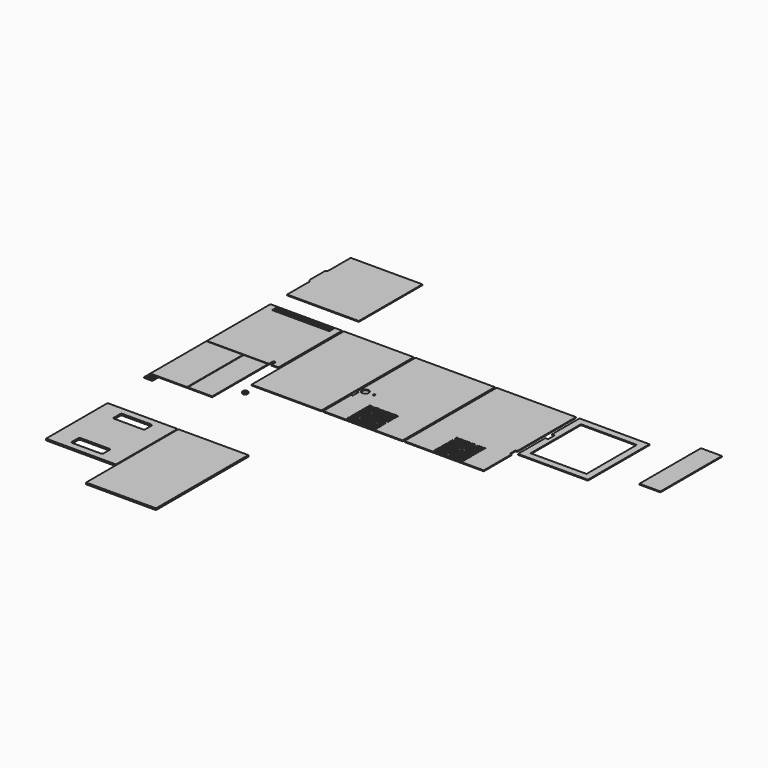
from build123d import *

# Parameters (mm, degrees)
F2_DEPTH  = 3.175
F1_W      = 38.1
F1_H      = 419.1
F1_W_2    = 215.9
F1_W_3    = 88.9
F1_H_2    = 254
F1_W_4    = 133.35
F1_R      = 9.3534635291
F1_R_2    = 1.5
F1_R_3    = 3.75
F1_W_5    = 6.35
F1_H_3    = 25.4
F1_W_6    = 203.2
F1_H_4    = 228.6
F1_W_7    = 76.2
F1_H_5    = 279.4
F4_W      = 254
F4_H      = 279.4
F4_W_2    = 114.3
F4_H_2    = 38.1
F5_DEPTH  = 5.9944
F4_H_3    = 419.1
F6_W      = 0.254
F6_H      = 88.9
F6_H_2    = 152.4
F7_DEPTH  = 0.508
F8_W      = 0.254
F8_H      = 88.9
F8_H_2    = 152.4
F9_DEPTH  = 0.508
F10_R     = 1.5875
F11_DEPTH = 5.9954
F14_DEPTH = 3.175
F15_R     = 3.75
F15_R_2   = 12.7
F16_DEPTH = 3.176
F17_R     = 5.08
F18_DEPTH = 5.9954


# Not quite as in the source:
# - a feature names something its author has since deleted; it is built from what else it names


with BuildPart() as f2:
    # F1 (on face) → F2 (new body)
    with BuildSketch(Plane.XY):
        with BuildLine():
            Line((-104.5470143864, 306.8558610559), (-364.8970143864, 306.8558610559))
            Line((-364.8970143864, 306.8558610559), (-364.8970143864, 18.2864610559))
            Line((-364.8970143864, 18.2864610559), (-139.4720143864, 18.2864610559))
            Line((-139.4720143864, 18.2864610559), (-139.4720143864, 34.1614610559))
            ThreePointArc((-139.4720143864, 34.1614610559), (-134.7095143864, 38.9239610559), (-129.9470143864, 34.1614610559))
            Line((-129.9470143864, 34.1614610559), (-129.9470143864, 18.2864610559))
            Line((-129.9470143864, 18.2864610559), (-104.5470143864, 18.2864610559))
            Line((-104.5470143864, 18.2864610559), (-104.5470143864, 306.8558610559))
        make_face()
        with BuildLine():
            ThreePointArc((-336.3220143864, 281.4558610559), (-339.4970143864, 284.6308610559), (-336.3220143864, 287.8058610559))
            Line((-336.3220143864, 287.8058610559), (-133.1220143864, 287.8058610559))
            ThreePointArc((-133.1220143864, 287.8058610559), (-129.9470143864, 284.6308610559), (-133.1220143864, 281.4558610559))
            Line((-133.1220143864, 281.4558610559), (-336.3220143864, 281.4558610559))
        make_face(mode=Mode.SUBTRACT)
        with BuildLine():
            ThreePointArc((-336.3220143864, 294.1558610559), (-339.4970143864, 297.3308610559), (-336.3220143864, 300.5058610559))
            Line((-336.3220143864, 300.5058610559), (-133.1220143864, 300.5058610559))
            ThreePointArc((-133.1220143864, 300.5058610559), (-129.9470143864, 297.3308610559), (-133.1220143864, 294.1558610559))
            Line((-133.1220143864, 294.1558610559), (-336.3220143864, 294.1558610559))
        make_face(mode=Mode.SUBTRACT)
    extrude(amount=F2_DEPTH)

    # F10 (on face) → F18 (cut, through all)
    with BuildSketch(Plane(origin=(0, 0, 0), x_dir=(1, 0, 0), z_dir=(0, 0, -1))):
        with Locations((244.9569856136, 4.2941389441)):
            Circle(F10_R)
        with Locations((244.9569856136, 10.6441389441)):
            Circle(F10_R)
        with Locations((244.9569856136, 16.9941389441)):
            Circle(F10_R)
        with Locations((244.9569856136, 23.3441389441)):
            Circle(F10_R)
        with Locations((244.9569856136, 29.6941389441)):
            Circle(F10_R)
        with Locations((244.9569856136, 36.0441389441)):
            Circle(F10_R)
        with Locations((244.9569856136, 42.3941389441)):
            Circle(F10_R)
        with Locations((244.9569856136, 48.7441389441)):
            Circle(F10_R)
        with Locations((244.9569856136, 55.0941389441)):
            Circle(F10_R)
        with Locations((244.9569856136, 61.4441389441)):
            Circle(F10_R)
        with Locations((244.9569856136, 67.7941389441)):
            Circle(F10_R)
        with Locations((244.9569856136, 74.1441389441)):
            Circle(F10_R)
        with Locations((244.9569856136, 80.4941389441)):
            Circle(F10_R)
        with Locations((244.9569856136, 86.8441389441)):
            Circle(F10_R)
        with Locations((244.9569856136, 93.1941389441)):
            Circle(F10_R)
        with Locations((244.9569856136, 99.5441389441)):
            Circle(F10_R)
        with Locations((244.9569856136, 105.8941389441)):
            Circle(F10_R)
        with Locations((251.3069856136, 4.2941389441)):
            Circle(F10_R)
        with Locations((251.3069856136, 10.6441389441)):
            Circle(F10_R)
        with Locations((251.3069856136, 16.9941389441)):
            Circle(F10_R)
        with Locations((251.3069856136, 23.3441389441)):
            Circle(F10_R)
        with Locations((251.3069856136, 29.6941389441)):
            Circle(F10_R)
        with Locations((251.3069856136, 36.0441389441)):
            Circle(F10_R)
        with Locations((251.3069856136, 42.3941389441)):
            Circle(F10_R)
        with Locations((251.3069856136, 48.7441389441)):
            Circle(F10_R)
        with Locations((251.3069856136, 55.0941389441)):
            Circle(F10_R)
        with Locations((251.3069856136, 61.4441389441)):
            Circle(F10_R)
        with Locations((251.3069856136, 67.7941389441)):
            Circle(F10_R)
        with Locations((251.3069856136, 74.1441389441)):
            Circle(F10_R)
        with Locations((251.3069856136, 80.4941389441)):
            Circle(F10_R)
        with Locations((251.3069856136, 86.8441389441)):
            Circle(F10_R)
        with Locations((251.3069856136, 93.1941389441)):
            Circle(F10_R)
        with Locations((251.3069856136, 99.5441389441)):
            Circle(F10_R)
        with Locations((251.3069856136, 105.8941389441)):
            Circle(F10_R)
        with Locations((257.6569856136, 4.2941389441)):
            Circle(F10_R)
        with Locations((257.6569856136, 10.6441389441)):
            Circle(F10_R)
        with Locations((257.6569856136, 16.9941389441)):
            Circle(F10_R)
        with Locations((257.6569856136, 23.3441389441)):
            Circle(F10_R)
        with Locations((257.6569856136, 29.6941389441)):
            Circle(F10_R)
        with Locations((257.6569856136, 36.0441389441)):
            Circle(F10_R)
        with Locations((257.6569856136, 42.3941389441)):
            Circle(F10_R)
        with Locations((257.6569856136, 48.7441389441)):
            Circle(F10_R)
        with Locations((257.6569856136, 55.0941389441)):
            Circle(F10_R)
        with Locations((257.6569856136, 61.4441389441)):
            Circle(F10_R)
        with Locations((257.6569856136, 67.7941389441)):
            Circle(F10_R)
        with Locations((257.6569856136, 74.1441389441)):
            Circle(F10_R)
        with Locations((257.6569856136, 80.4941389441)):
            Circle(F10_R)
        with Locations((257.6569856136, 86.8441389441)):
            Circle(F10_R)
        with Locations((257.6569856136, 93.1941389441)):
            Circle(F10_R)
        with Locations((257.6569856136, 99.5441389441)):
            Circle(F10_R)
        with Locations((257.6569856136, 105.8941389441)):
            Circle(F10_R)
        with Locations((264.0069856136, 4.2941389441)):
            Circle(F10_R)
        with Locations((264.0069856136, 10.6441389441)):
            Circle(F10_R)
        with Locations((264.0069856136, 16.9941389441)):
            Circle(F10_R)
        with Locations((264.0069856136, 23.3441389441)):
            Circle(F10_R)
        with Locations((264.0069856136, 29.6941389441)):
            Circle(F10_R)
        with Locations((264.0069856136, 36.0441389441)):
            Circle(F10_R)
        with Locations((264.0069856136, 42.3941389441)):
            Circle(F10_R)
        with Locations((264.0069856136, 48.7441389441)):
            Circle(F10_R)
        with Locations((264.0069856136, 55.0941389441)):
            Circle(F10_R)
        with Locations((264.0069856136, 61.4441389441)):
            Circle(F10_R)
        with Locations((264.0069856136, 67.7941389441)):
            Circle(F10_R)
        with Locations((264.0069856136, 74.1441389441)):
            Circle(F10_R)
        with Locations((264.0069856136, 80.4941389441)):
            Circle(F10_R)
        with Locations((264.0069856136, 86.8441389441)):
            Circle(F10_R)
        with Locations((264.0069856136, 93.1941389441)):
            Circle(F10_R)
        with Locations((264.0069856136, 99.5441389441)):
            Circle(F10_R)
        with Locations((264.0069856136, 105.8941389441)):
            Circle(F10_R)
        with Locations((270.3569856136, 4.2941389441)):
            Circle(F10_R)
        with Locations((270.3569856136, 10.6441389441)):
            Circle(F10_R)
        with Locations((270.3569856136, 16.9941389441)):
            Circle(F10_R)
        with Locations((270.3569856136, 23.3441389441)):
            Circle(F10_R)
        with Locations((270.3569856136, 29.6941389441)):
            Circle(F10_R)
        with Locations((270.3569856136, 36.0441389441)):
            Circle(F10_R)
        with Locations((270.3569856136, 42.3941389441)):
            Circle(F10_R)
        with Locations((270.3569856136, 48.7441389441)):
            Circle(F10_R)
        with Locations((270.3569856136, 55.0941389441)):
            Circle(F10_R)
        with Locations((270.3569856136, 61.4441389441)):
            Circle(F10_R)
        with Locations((270.3569856136, 67.7941389441)):
            Circle(F10_R)
        with Locations((270.3569856136, 74.1441389441)):
            Circle(F10_R)
        with Locations((270.3569856136, 80.4941389441)):
            Circle(F10_R)
        with Locations((270.3569856136, 86.8441389441)):
            Circle(F10_R)
        with Locations((270.3569856136, 93.1941389441)):
            Circle(F10_R)
        with Locations((270.3569856136, 99.5441389441)):
            Circle(F10_R)
        with Locations((270.3569856136, 105.8941389441)):
            Circle(F10_R)
        with Locations((276.7069856136, 4.2941389441)):
            Circle(F10_R)
        with Locations((276.7069856136, 10.6441389441)):
            Circle(F10_R)
        with Locations((276.7069856136, 16.9941389441)):
            Circle(F10_R)
        with Locations((276.7069856136, 23.3441389441)):
            Circle(F10_R)
        with Locations((276.7069856136, 29.6941389441)):
            Circle(F10_R)
        with Locations((276.7069856136, 36.0441389441)):
            Circle(F10_R)
        with Locations((276.7069856136, 42.3941389441)):
            Circle(F10_R)
        with Locations((276.7069856136, 48.7441389441)):
            Circle(F10_R)
        with Locations((276.7069856136, 55.0941389441)):
            Circle(F10_R)
        with Locations((276.7069856136, 61.4441389441)):
            Circle(F10_R)
        with Locations((276.7069856136, 67.7941389441)):
            Circle(F10_R)
        with Locations((276.7069856136, 74.1441389441)):
            Circle(F10_R)
        with Locations((276.7069856136, 80.4941389441)):
            Circle(F10_R)
        with Locations((276.7069856136, 86.8441389441)):
            Circle(F10_R)
        with Locations((276.7069856136, 93.1941389441)):
            Circle(F10_R)
        with Locations((276.7069856136, 99.5441389441)):
            Circle(F10_R)
        with Locations((276.7069856136, 105.8941389441)):
            Circle(F10_R)
        with Locations((283.0569856136, 4.2941389441)):
            Circle(F10_R)
        with Locations((283.0569856136, 10.6441389441)):
            Circle(F10_R)
        with Locations((283.0569856136, 16.9941389441)):
            Circle(F10_R)
        with Locations((283.0569856136, 23.3441389441)):
            Circle(F10_R)
        with Locations((283.0569856136, 29.6941389441)):
            Circle(F10_R)
        with Locations((283.0569856136, 36.0441389441)):
            Circle(F10_R)
        with Locations((283.0569856136, 42.3941389441)):
            Circle(F10_R)
        with Locations((283.0569856136, 48.7441389441)):
            Circle(F10_R)
        with Locations((283.0569856136, 55.0941389441)):
            Circle(F10_R)
        with Locations((283.0569856136, 61.4441389441)):
            Circle(F10_R)
        with Locations((283.0569856136, 67.7941389441)):
            Circle(F10_R)
        with Locations((283.0569856136, 74.1441389441)):
            Circle(F10_R)
        with Locations((283.0569856136, 80.4941389441)):
            Circle(F10_R)
        with Locations((283.0569856136, 86.8441389441)):
            Circle(F10_R)
        with Locations((283.0569856136, 93.1941389441)):
            Circle(F10_R)
        with Locations((283.0569856136, 99.5441389441)):
            Circle(F10_R)
        with Locations((283.0569856136, 105.8941389441)):
            Circle(F10_R)
        with Locations((289.4069856136, 4.2941389441)):
            Circle(F10_R)
        with Locations((289.4069856136, 10.6441389441)):
            Circle(F10_R)
        with Locations((289.4069856136, 16.9941389441)):
            Circle(F10_R)
        with Locations((289.4069856136, 23.3441389441)):
            Circle(F10_R)
        with Locations((289.4069856136, 29.6941389441)):
            Circle(F10_R)
        with Locations((289.4069856136, 36.0441389441)):
            Circle(F10_R)
        with Locations((289.4069856136, 42.3941389441)):
            Circle(F10_R)
        with Locations((289.4069856136, 48.7441389441)):
            Circle(F10_R)
        with Locations((289.4069856136, 55.0941389441)):
            Circle(F10_R)
        with Locations((289.4069856136, 61.4441389441)):
            Circle(F10_R)
        with Locations((289.4069856136, 67.7941389441)):
            Circle(F10_R)
        with Locations((289.4069856136, 74.1441389441)):
            Circle(F10_R)
        with Locations((289.4069856136, 80.4941389441)):
            Circle(F10_R)
        with Locations((289.4069856136, 86.8441389441)):
            Circle(F10_R)
        with Locations((289.4069856136, 93.1941389441)):
            Circle(F10_R)
        with Locations((289.4069856136, 99.5441389441)):
            Circle(F10_R)
        with Locations((289.4069856136, 105.8941389441)):
            Circle(F10_R)
        with Locations((295.7569856136, 4.2941389441)):
            Circle(F10_R)
        with Locations((295.7569856136, 10.6441389441)):
            Circle(F10_R)
        with Locations((295.7569856136, 16.9941389441)):
            Circle(F10_R)
        with Locations((295.7569856136, 23.3441389441)):
            Circle(F10_R)
        with Locations((295.7569856136, 29.6941389441)):
            Circle(F10_R)
        with Locations((295.7569856136, 36.0441389441)):
            Circle(F10_R)
        with Locations((295.7569856136, 42.3941389441)):
            Circle(F10_R)
        with Locations((295.7569856136, 48.7441389441)):
            Circle(F10_R)
        with Locations((295.7569856136, 55.0941389441)):
            Circle(F10_R)
        with Locations((295.7569856136, 61.4441389441)):
            Circle(F10_R)
        with Locations((295.7569856136, 67.7941389441)):
            Circle(F10_R)
        with Locations((295.7569856136, 74.1441389441)):
            Circle(F10_R)
        with Locations((295.7569856136, 80.4941389441)):
            Circle(F10_R)
        with Locations((295.7569856136, 86.8441389441)):
            Circle(F10_R)
        with Locations((295.7569856136, 93.1941389441)):
            Circle(F10_R)
        with Locations((295.7569856136, 99.5441389441)):
            Circle(F10_R)
        with Locations((295.7569856136, 105.8941389441)):
            Circle(F10_R)
        with Locations((302.1069856136, 4.2941389441)):
            Circle(F10_R)
        with Locations((302.1069856136, 10.6441389441)):
            Circle(F10_R)
        with Locations((302.1069856136, 16.9941389441)):
            Circle(F10_R)
        with Locations((302.1069856136, 23.3441389441)):
            Circle(F10_R)
        with Locations((302.1069856136, 29.6941389441)):
            Circle(F10_R)
        with Locations((302.1069856136, 36.0441389441)):
            Circle(F10_R)
        with Locations((302.1069856136, 42.3941389441)):
            Circle(F10_R)
        with Locations((302.1069856136, 48.7441389441)):
            Circle(F10_R)
        with Locations((302.1069856136, 55.0941389441)):
            Circle(F10_R)
        with Locations((302.1069856136, 61.4441389441)):
            Circle(F10_R)
        with Locations((302.1069856136, 67.7941389441)):
            Circle(F10_R)
        with Locations((302.1069856136, 74.1441389441)):
            Circle(F10_R)
        with Locations((302.1069856136, 80.4941389441)):
            Circle(F10_R)
        with Locations((302.1069856136, 86.8441389441)):
            Circle(F10_R)
        with Locations((302.1069856136, 93.1941389441)):
            Circle(F10_R)
        with Locations((302.1069856136, 99.5441389441)):
            Circle(F10_R)
        with Locations((302.1069856136, 105.8941389441)):
            Circle(F10_R)
        with Locations((308.4569856136, 4.2941389441)):
            Circle(F10_R)
        with Locations((308.4569856136, 10.6441389441)):
            Circle(F10_R)
        with Locations((308.4569856136, 16.9941389441)):
            Circle(F10_R)
        with Locations((308.4569856136, 23.3441389441)):
            Circle(F10_R)
        with Locations((308.4569856136, 29.6941389441)):
            Circle(F10_R)
        with Locations((308.4569856136, 36.0441389441)):
            Circle(F10_R)
        with Locations((308.4569856136, 42.3941389441)):
            Circle(F10_R)
        with Locations((308.4569856136, 48.7441389441)):
            Circle(F10_R)
        with Locations((308.4569856136, 55.0941389441)):
            Circle(F10_R)
        with Locations((308.4569856136, 61.4441389441)):
            Circle(F10_R)
        with Locations((308.4569856136, 67.7941389441)):
            Circle(F10_R)
        with Locations((308.4569856136, 74.1441389441)):
            Circle(F10_R)
        with Locations((308.4569856136, 80.4941389441)):
            Circle(F10_R)
        with Locations((308.4569856136, 86.8441389441)):
            Circle(F10_R)
        with Locations((308.4569856136, 93.1941389441)):
            Circle(F10_R)
        with Locations((308.4569856136, 99.5441389441)):
            Circle(F10_R)
        with Locations((308.4569856136, 105.8941389441)):
            Circle(F10_R)
        with Locations((314.8069856136, 4.2941389441)):
            Circle(F10_R)
        with Locations((314.8069856136, 10.6441389441)):
            Circle(F10_R)
        with Locations((314.8069856136, 16.9941389441)):
            Circle(F10_R)
        with Locations((314.8069856136, 23.3441389441)):
            Circle(F10_R)
        with Locations((314.8069856136, 29.6941389441)):
            Circle(F10_R)
        with Locations((314.8069856136, 36.0441389441)):
            Circle(F10_R)
        with Locations((314.8069856136, 42.3941389441)):
            Circle(F10_R)
        with Locations((314.8069856136, 48.7441389441)):
            Circle(F10_R)
        with Locations((314.8069856136, 55.0941389441)):
            Circle(F10_R)
        with Locations((314.8069856136, 61.4441389441)):
            Circle(F10_R)
        with Locations((314.8069856136, 67.7941389441)):
            Circle(F10_R)
        with Locations((314.8069856136, 74.1441389441)):
            Circle(F10_R)
        with Locations((314.8069856136, 80.4941389441)):
            Circle(F10_R)
        with Locations((314.8069856136, 86.8441389441)):
            Circle(F10_R)
        with Locations((314.8069856136, 93.1941389441)):
            Circle(F10_R)
        with Locations((314.8069856136, 99.5441389441)):
            Circle(F10_R)
        with Locations((314.8069856136, 105.8941389441)):
            Circle(F10_R)
        with Locations((321.1569856136, 4.2941389441)):
            Circle(F10_R)
        with Locations((321.1569856136, 10.6441389441)):
            Circle(F10_R)
        with Locations((321.1569856136, 16.9941389441)):
            Circle(F10_R)
        with Locations((321.1569856136, 23.3441389441)):
            Circle(F10_R)
        with Locations((321.1569856136, 29.6941389441)):
            Circle(F10_R)
        with Locations((321.1569856136, 36.0441389441)):
            Circle(F10_R)
        with Locations((321.1569856136, 42.3941389441)):
            Circle(F10_R)
        with Locations((321.1569856136, 48.7441389441)):
            Circle(F10_R)
        with Locations((321.1569856136, 55.0941389441)):
            Circle(F10_R)
        with Locations((321.1569856136, 61.4441389441)):
            Circle(F10_R)
        with Locations((321.1569856136, 67.7941389441)):
            Circle(F10_R)
        with Locations((321.1569856136, 74.1441389441)):
            Circle(F10_R)
        with Locations((321.1569856136, 80.4941389441)):
            Circle(F10_R)
        with Locations((321.1569856136, 86.8441389441)):
            Circle(F10_R)
        with Locations((321.1569856136, 93.1941389441)):
            Circle(F10_R)
        with Locations((321.1569856136, 99.5441389441)):
            Circle(F10_R)
        with Locations((321.1569856136, 105.8941389441)):
            Circle(F10_R)
        with Locations((327.5069856136, 4.2941389441)):
            Circle(F10_R)
        with Locations((327.5069856136, 10.6441389441)):
            Circle(F10_R)
        with Locations((327.5069856136, 16.9941389441)):
            Circle(F10_R)
        with Locations((327.5069856136, 23.3441389441)):
            Circle(F10_R)
        with Locations((327.5069856136, 29.6941389441)):
            Circle(F10_R)
        with Locations((327.5069856136, 36.0441389441)):
            Circle(F10_R)
        with Locations((327.5069856136, 42.3941389441)):
            Circle(F10_R)
        with Locations((327.5069856136, 48.7441389441)):
            Circle(F10_R)
        with Locations((327.5069856136, 55.0941389441)):
            Circle(F10_R)
        with Locations((327.5069856136, 61.4441389441)):
            Circle(F10_R)
        with Locations((327.5069856136, 67.7941389441)):
            Circle(F10_R)
        with Locations((327.5069856136, 74.1441389441)):
            Circle(F10_R)
        with Locations((327.5069856136, 80.4941389441)):
            Circle(F10_R)
        with Locations((327.5069856136, 86.8441389441)):
            Circle(F10_R)
        with Locations((327.5069856136, 93.1941389441)):
            Circle(F10_R)
        with Locations((327.5069856136, 99.5441389441)):
            Circle(F10_R)
        with Locations((327.5069856136, 105.8941389441)):
            Circle(F10_R)
        with Locations((333.8569856136, 4.2941389441)):
            Circle(F10_R)
        with Locations((333.8569856136, 10.6441389441)):
            Circle(F10_R)
        with Locations((333.8569856136, 16.9941389441)):
            Circle(F10_R)
        with Locations((333.8569856136, 23.3441389441)):
            Circle(F10_R)
        with Locations((333.8569856136, 29.6941389441)):
            Circle(F10_R)
        with Locations((333.8569856136, 36.0441389441)):
            Circle(F10_R)
        with Locations((333.8569856136, 42.3941389441)):
            Circle(F10_R)
        with Locations((333.8569856136, 48.7441389441)):
            Circle(F10_R)
        with Locations((333.8569856136, 55.0941389441)):
            Circle(F10_R)
        with Locations((333.8569856136, 61.4441389441)):
            Circle(F10_R)
        with Locations((333.8569856136, 67.7941389441)):
            Circle(F10_R)
        with Locations((333.8569856136, 74.1441389441)):
            Circle(F10_R)
        with Locations((333.8569856136, 80.4941389441)):
            Circle(F10_R)
        with Locations((333.8569856136, 86.8441389441)):
            Circle(F10_R)
        with Locations((333.8569856136, 93.1941389441)):
            Circle(F10_R)
        with Locations((333.8569856136, 99.5441389441)):
            Circle(F10_R)
        with Locations((333.8569856136, 105.8941389441)):
            Circle(F10_R)
        with Locations((340.2069856136, 4.2941389441)):
            Circle(F10_R)
        with Locations((340.2069856136, 10.6441389441)):
            Circle(F10_R)
        with Locations((340.2069856136, 16.9941389441)):
            Circle(F10_R)
        with Locations((340.2069856136, 23.3441389441)):
            Circle(F10_R)
        with Locations((340.2069856136, 29.6941389441)):
            Circle(F10_R)
        with Locations((340.2069856136, 36.0441389441)):
            Circle(F10_R)
        with Locations((340.2069856136, 42.3941389441)):
            Circle(F10_R)
        with Locations((340.2069856136, 48.7441389441)):
            Circle(F10_R)
        with Locations((340.2069856136, 55.0941389441)):
            Circle(F10_R)
        with Locations((340.2069856136, 61.4441389441)):
            Circle(F10_R)
        with Locations((340.2069856136, 67.7941389441)):
            Circle(F10_R)
        with Locations((340.2069856136, 74.1441389441)):
            Circle(F10_R)
        with Locations((340.2069856136, 80.4941389441)):
            Circle(F10_R)
        with Locations((340.2069856136, 86.8441389441)):
            Circle(F10_R)
        with Locations((340.2069856136, 93.1941389441)):
            Circle(F10_R)
        with Locations((340.2069856136, 99.5441389441)):
            Circle(F10_R)
        with Locations((340.2069856136, 105.8941389441)):
            Circle(F10_R)
        with Locations((346.5569856136, 4.2941389441)):
            Circle(F10_R)
        with Locations((346.5569856136, 10.6441389441)):
            Circle(F10_R)
        with Locations((346.5569856136, 16.9941389441)):
            Circle(F10_R)
        with Locations((346.5569856136, 23.3441389441)):
            Circle(F10_R)
        with Locations((346.5569856136, 29.6941389441)):
            Circle(F10_R)
        with Locations((346.5569856136, 36.0441389441)):
            Circle(F10_R)
        with Locations((346.5569856136, 42.3941389441)):
            Circle(F10_R)
        with Locations((346.5569856136, 48.7441389441)):
            Circle(F10_R)
        with Locations((346.5569856136, 55.0941389441)):
            Circle(F10_R)
        with Locations((346.5569856136, 61.4441389441)):
            Circle(F10_R)
        with Locations((346.5569856136, 67.7941389441)):
            Circle(F10_R)
        with Locations((346.5569856136, 74.1441389441)):
            Circle(F10_R)
        with Locations((346.5569856136, 80.4941389441)):
            Circle(F10_R)
        with Locations((346.5569856136, 86.8441389441)):
            Circle(F10_R)
        with Locations((346.5569856136, 93.1941389441)):
            Circle(F10_R)
        with Locations((346.5569856136, 99.5441389441)):
            Circle(F10_R)
        with Locations((346.5569856136, 105.8941389441)):
            Circle(F10_R)
        with Locations((662.8377856136, 4.2941389441)):
            Circle(F10_R)
        with Locations((561.2377856136, 105.8941389441)):
            Circle(F10_R)
        with Locations((662.8377856136, 105.8941389441)):
            Circle(F10_R)
        with Locations((561.2377856136, 4.2941389441)):
            Circle(F10_R)
        with Locations((656.4877856136, 4.2941389441)):
            Circle(F10_R)
        with Locations((662.8377856136, 10.6441389441)):
            Circle(F10_R)
        with Locations((612.0377856136, 48.7441389441)):
            Circle(F10_R)
        with Locations((618.3877856136, 10.6441389441)):
            Circle(F10_R)
        with Locations((618.3877856136, 99.5441389441)):
            Circle(F10_R)
        with Locations((618.3877856136, 55.0941389441)):
            Circle(F10_R)
        with Locations((567.5877856136, 16.9941389441)):
            Circle(F10_R)
        with Locations((650.1377856136, 61.4441389441)):
            Circle(F10_R)
        with Locations((586.6377856136, 80.4941389441)):
            Circle(F10_R)
        with Locations((618.3877856136, 105.8941389441)):
            Circle(F10_R)
        with Locations((599.3377856136, 93.1941389441)):
            Circle(F10_R)
        with Locations((605.6877856136, 74.1441389441)):
            Circle(F10_R)
        with Locations((573.9377856136, 93.1941389441)):
            Circle(F10_R)
        with Locations((573.9377856136, 67.7941389441)):
            Circle(F10_R)
        with Locations((599.3377856136, 10.6441389441)):
            Circle(F10_R)
        with Locations((643.7877856136, 4.2941389441)):
            Circle(F10_R)
        with Locations((567.5877856136, 42.3941389441)):
            Circle(F10_R)
        with Locations((656.4877856136, 99.5441389441)):
            Circle(F10_R)
        with Locations((656.4877856136, 42.3941389441)):
            Circle(F10_R)
        with Locations((643.7877856136, 86.8441389441)):
            Circle(F10_R)
        with Locations((662.8377856136, 86.8441389441)):
            Circle(F10_R)
        with Locations((662.8377856136, 74.1441389441)):
            Circle(F10_R)
        with Locations((650.1377856136, 36.0441389441)):
            Circle(F10_R)
        with Locations((637.4377856136, 16.9941389441)):
            Circle(F10_R)
        with Locations((624.7377856136, 36.0441389441)):
            Circle(F10_R)
        with Locations((662.8377856136, 23.3441389441)):
            Circle(F10_R)
        with Locations((592.9877856136, 29.6941389441)):
            Circle(F10_R)
        with Locations((618.3877856136, 93.1941389441)):
            Circle(F10_R)
        with Locations((624.7377856136, 61.4441389441)):
            Circle(F10_R)
        with Locations((592.9877856136, 61.4441389441)):
            Circle(F10_R)
        with Locations((612.0377856136, 80.4941389441)):
            Circle(F10_R)
        with Locations((586.6377856136, 55.0941389441)):
            Circle(F10_R)
        with Locations((605.6877856136, 105.8941389441)):
            Circle(F10_R)
        with Locations((612.0377856136, 36.0441389441)):
            Circle(F10_R)
        with Locations((561.2377856136, 86.8441389441)):
            Circle(F10_R)
        with Locations((599.3377856136, 16.9941389441)):
            Circle(F10_R)
        with Locations((624.7377856136, 42.3941389441)):
            Circle(F10_R)
        with Locations((561.2377856136, 67.7941389441)):
            Circle(F10_R)
        with Locations((637.4377856136, 80.4941389441)):
            Circle(F10_R)
        with Locations((637.4377856136, 36.0441389441)):
            Circle(F10_R)
        with Locations((561.2377856136, 16.9941389441)):
            Circle(F10_R)
        with Locations((656.4877856136, 10.6441389441)):
            Circle(F10_R)
        with Locations((605.6877856136, 23.3441389441)):
            Circle(F10_R)
        with Locations((580.2877856136, 16.9941389441)):
            Circle(F10_R)
        with Locations((599.3377856136, 67.7941389441)):
            Circle(F10_R)
        with Locations((656.4877856136, 80.4941389441)):
            Circle(F10_R)
        with Locations((573.9377856136, 74.1441389441)):
            Circle(F10_R)
        with Locations((650.1377856136, 74.1441389441)):
            Circle(F10_R)
        with Locations((567.5877856136, 10.6441389441)):
            Circle(F10_R)
        with Locations((650.1377856136, 42.3941389441)):
            Circle(F10_R)
        with Locations((586.6377856136, 48.7441389441)):
            Circle(F10_R)
        with Locations((618.3877856136, 48.7441389441)):
            Circle(F10_R)
        with Locations((656.4877856136, 67.7941389441)):
            Circle(F10_R)
        with Locations((567.5877856136, 36.0441389441)):
            Circle(F10_R)
        with Locations((624.7377856136, 23.3441389441)):
            Circle(F10_R)
        with Locations((567.5877856136, 23.3441389441)):
            Circle(F10_R)
        with Locations((618.3877856136, 4.2941389441)):
            Circle(F10_R)
        with Locations((637.4377856136, 99.5441389441)):
            Circle(F10_R)
        with Locations((592.9877856136, 93.1941389441)):
            Circle(F10_R)
        with Locations((561.2377856136, 48.7441389441)):
            Circle(F10_R)
        with Locations((637.4377856136, 61.4441389441)):
            Circle(F10_R)
        with Locations((567.5877856136, 29.6941389441)):
            Circle(F10_R)
        with Locations((592.9877856136, 23.3441389441)):
            Circle(F10_R)
        with Locations((650.1377856136, 23.3441389441)):
            Circle(F10_R)
        with Locations((631.0877856136, 36.0441389441)):
            Circle(F10_R)
        with Locations((580.2877856136, 80.4941389441)):
            Circle(F10_R)
        with Locations((605.6877856136, 4.2941389441)):
            Circle(F10_R)
        with Locations((631.0877856136, 16.9941389441)):
            Circle(F10_R)
        with Locations((650.1377856136, 16.9941389441)):
            Circle(F10_R)
        with Locations((605.6877856136, 10.6441389441)):
            Circle(F10_R)
        with Locations((592.9877856136, 74.1441389441)):
            Circle(F10_R)
        with Locations((605.6877856136, 61.4441389441)):
            Circle(F10_R)
        with Locations((637.4377856136, 10.6441389441)):
            Circle(F10_R)
        with Locations((586.6377856136, 42.3941389441)):
            Circle(F10_R)
        with Locations((580.2877856136, 10.6441389441)):
            Circle(F10_R)
        with Locations((561.2377856136, 10.6441389441)):
            Circle(F10_R)
        with Locations((643.7877856136, 93.1941389441)):
            Circle(F10_R)
        with Locations((573.9377856136, 86.8441389441)):
            Circle(F10_R)
        with Locations((561.2377856136, 23.3441389441)):
            Circle(F10_R)
        with Locations((618.3877856136, 36.0441389441)):
            Circle(F10_R)
        with Locations((573.9377856136, 42.3941389441)):
            Circle(F10_R)
        with Locations((631.0877856136, 105.8941389441)):
            Circle(F10_R)
        with Locations((631.0877856136, 29.6941389441)):
            Circle(F10_R)
        with Locations((643.7877856136, 61.4441389441)):
            Circle(F10_R)
        with Locations((612.0377856136, 74.1441389441)):
            Circle(F10_R)
        with Locations((599.3377856136, 80.4941389441)):
            Circle(F10_R)
        with Locations((631.0877856136, 61.4441389441)):
            Circle(F10_R)
        with Locations((618.3877856136, 23.3441389441)):
            Circle(F10_R)
        with Locations((580.2877856136, 36.0441389441)):
            Circle(F10_R)
        with Locations((656.4877856136, 36.0441389441)):
            Circle(F10_R)
        with Locations((662.8377856136, 36.0441389441)):
            Circle(F10_R)
        with Locations((643.7877856136, 48.7441389441)):
            Circle(F10_R)
        with Locations((662.8377856136, 48.7441389441)):
            Circle(F10_R)
        with Locations((599.3377856136, 42.3941389441)):
            Circle(F10_R)
        with Locations((650.1377856136, 29.6941389441)):
            Circle(F10_R)
        with Locations((586.6377856136, 10.6441389441)):
            Circle(F10_R)
        with Locations((631.0877856136, 67.7941389441)):
            Circle(F10_R)
        with Locations((605.6877856136, 55.0941389441)):
            Circle(F10_R)
        with Locations((580.2877856136, 86.8441389441)):
            Circle(F10_R)
        with Locations((599.3377856136, 4.2941389441)):
            Circle(F10_R)
        with Locations((592.9877856136, 67.7941389441)):
            Circle(F10_R)
        with Locations((643.7877856136, 105.8941389441)):
            Circle(F10_R)
        with Locations((580.2877856136, 105.8941389441)):
            Circle(F10_R)
        with Locations((573.9377856136, 99.5441389441)):
            Circle(F10_R)
        with Locations((561.2377856136, 93.1941389441)):
            Circle(F10_R)
        with Locations((580.2877856136, 23.3441389441)):
            Circle(F10_R)
        with Locations((573.9377856136, 16.9941389441)):
            Circle(F10_R)
        with Locations((650.1377856136, 99.5441389441)):
            Circle(F10_R)
        with Locations((650.1377856136, 4.2941389441)):
            Circle(F10_R)
        with Locations((586.6377856136, 93.1941389441)):
            Circle(F10_R)
        with Locations((662.8377856136, 42.3941389441)):
            Circle(F10_R)
        with Locations((631.0877856136, 23.3441389441)):
            Circle(F10_R)
        with Locations((618.3877856136, 67.7941389441)):
            Circle(F10_R)
        with Locations((592.9877856136, 99.5441389441)):
            Circle(F10_R)
        with Locations((643.7877856136, 16.9941389441)):
            Circle(F10_R)
        with Locations((631.0877856136, 48.7441389441)):
            Circle(F10_R)
        with Locations((643.7877856136, 36.0441389441)):
            Circle(F10_R)
        with Locations((612.0377856136, 86.8441389441)):
            Circle(F10_R)
        with Locations((637.4377856136, 86.8441389441)):
            Circle(F10_R)
        with Locations((612.0377856136, 99.5441389441)):
            Circle(F10_R)
        with Locations((605.6877856136, 42.3941389441)):
            Circle(F10_R)
        with Locations((624.7377856136, 93.1941389441)):
            Circle(F10_R)
        with Locations((567.5877856136, 67.7941389441)):
            Circle(F10_R)
        with Locations((605.6877856136, 48.7441389441)):
            Circle(F10_R)
        with Locations((573.9377856136, 29.6941389441)):
            Circle(F10_R)
        with Locations((561.2377856136, 74.1441389441)):
            Circle(F10_R)
        with Locations((637.4377856136, 23.3441389441)):
            Circle(F10_R)
        with Locations((637.4377856136, 29.6941389441)):
            Circle(F10_R)
        with Locations((624.7377856136, 86.8441389441)):
            Circle(F10_R)
        with Locations((580.2877856136, 67.7941389441)):
            Circle(F10_R)
        with Locations((586.6377856136, 105.8941389441)):
            Circle(F10_R)
        with Locations((586.6377856136, 16.9941389441)):
            Circle(F10_R)
        with Locations((662.8377856136, 80.4941389441)):
            Circle(F10_R)
        with Locations((580.2877856136, 42.3941389441)):
            Circle(F10_R)
        with Locations((592.9877856136, 10.6441389441)):
            Circle(F10_R)
        with Locations((618.3877856136, 86.8441389441)):
            Circle(F10_R)
        with Locations((561.2377856136, 42.3941389441)):
            Circle(F10_R)
        with Locations((567.5877856136, 105.8941389441)):
            Circle(F10_R)
        with Locations((643.7877856136, 55.0941389441)):
            Circle(F10_R)
        with Locations((592.9877856136, 55.0941389441)):
            Circle(F10_R)
        with Locations((599.3377856136, 48.7441389441)):
            Circle(F10_R)
        with Locations((624.7377856136, 16.9941389441)):
            Circle(F10_R)
        with Locations((643.7877856136, 23.3441389441)):
            Circle(F10_R)
        with Locations((573.9377856136, 55.0941389441)):
            Circle(F10_R)
        with Locations((586.6377856136, 29.6941389441)):
            Circle(F10_R)
        with Locations((592.9877856136, 80.4941389441)):
            Circle(F10_R)
        with Locations((650.1377856136, 48.7441389441)):
            Circle(F10_R)
        with Locations((605.6877856136, 86.8441389441)):
            Circle(F10_R)
        with Locations((592.9877856136, 16.9941389441)):
            Circle(F10_R)
        with Locations((643.7877856136, 42.3941389441)):
            Circle(F10_R)
        with Locations((567.5877856136, 61.4441389441)):
            Circle(F10_R)
        with Locations((605.6877856136, 16.9941389441)):
            Circle(F10_R)
        with Locations((656.4877856136, 86.8441389441)):
            Circle(F10_R)
        with Locations((618.3877856136, 61.4441389441)):
            Circle(F10_R)
        with Locations((605.6877856136, 29.6941389441)):
            Circle(F10_R)
        with Locations((561.2377856136, 99.5441389441)):
            Circle(F10_R)
        with Locations((618.3877856136, 74.1441389441)):
            Circle(F10_R)
        with Locations((592.9877856136, 36.0441389441)):
            Circle(F10_R)
        with Locations((656.4877856136, 16.9941389441)):
            Circle(F10_R)
        with Locations((586.6377856136, 99.5441389441)):
            Circle(F10_R)
        with Locations((599.3377856136, 55.0941389441)):
            Circle(F10_R)
        with Locations((656.4877856136, 61.4441389441)):
            Circle(F10_R)
        with Locations((637.4377856136, 74.1441389441)):
            Circle(F10_R)
        with Locations((573.9377856136, 105.8941389441)):
            Circle(F10_R)
        with Locations((624.7377856136, 105.8941389441)):
            Circle(F10_R)
        with Locations((624.7377856136, 29.6941389441)):
            Circle(F10_R)
        with Locations((586.6377856136, 61.4441389441)):
            Circle(F10_R)
        with Locations((631.0877856136, 10.6441389441)):
            Circle(F10_R)
        with Locations((586.6377856136, 74.1441389441)):
            Circle(F10_R)
        with Locations((612.0377856136, 23.3441389441)):
            Circle(F10_R)
        with Locations((656.4877856136, 105.8941389441)):
            Circle(F10_R)
        with Locations((650.1377856136, 67.7941389441)):
            Circle(F10_R)
        with Locations((605.6877856136, 99.5441389441)):
            Circle(F10_R)
        with Locations((567.5877856136, 99.5441389441)):
            Circle(F10_R)
        with Locations((662.8377856136, 93.1941389441)):
            Circle(F10_R)
        with Locations((650.1377856136, 86.8441389441)):
            Circle(F10_R)
        with Locations((605.6877856136, 36.0441389441)):
            Circle(F10_R)
        with Locations((618.3877856136, 16.9941389441)):
            Circle(F10_R)
        with Locations((580.2877856136, 93.1941389441)):
            Circle(F10_R)
        with Locations((586.6377856136, 36.0441389441)):
            Circle(F10_R)
        with Locations((561.2377856136, 80.4941389441)):
            Circle(F10_R)
        with Locations((637.4377856136, 42.3941389441)):
            Circle(F10_R)
        with Locations((631.0877856136, 42.3941389441)):
            Circle(F10_R)
        with Locations((662.8377856136, 61.4441389441)):
            Circle(F10_R)
        with Locations((573.9377856136, 36.0441389441)):
            Circle(F10_R)
        with Locations((612.0377856136, 16.9941389441)):
            Circle(F10_R)
        with Locations((567.5877856136, 74.1441389441)):
            Circle(F10_R)
        with Locations((631.0877856136, 55.0941389441)):
            Circle(F10_R)
        with Locations((631.0877856136, 80.4941389441)):
            Circle(F10_R)
        with Locations((637.4377856136, 48.7441389441)):
            Circle(F10_R)
        with Locations((662.8377856136, 29.6941389441)):
            Circle(F10_R)
        with Locations((586.6377856136, 67.7941389441)):
            Circle(F10_R)
        with Locations((650.1377856136, 93.1941389441)):
            Circle(F10_R)
        with Locations((592.9877856136, 48.7441389441)):
            Circle(F10_R)
        with Locations((586.6377856136, 86.8441389441)):
            Circle(F10_R)
        with Locations((631.0877856136, 74.1441389441)):
            Circle(F10_R)
        with Locations((580.2877856136, 48.7441389441)):
            Circle(F10_R)
        with Locations((612.0377856136, 55.0941389441)):
            Circle(F10_R)
        with Locations((612.0377856136, 29.6941389441)):
            Circle(F10_R)
        with Locations((612.0377856136, 105.8941389441)):
            Circle(F10_R)
        with Locations((573.9377856136, 48.7441389441)):
            Circle(F10_R)
        with Locations((599.3377856136, 74.1441389441)):
            Circle(F10_R)
        with Locations((605.6877856136, 67.7941389441)):
            Circle(F10_R)
        with Locations((561.2377856136, 61.4441389441)):
            Circle(F10_R)
        with Locations((643.7877856136, 67.7941389441)):
            Circle(F10_R)
        with Locations((567.5877856136, 80.4941389441)):
            Circle(F10_R)
        with Locations((624.7377856136, 67.7941389441)):
            Circle(F10_R)
        with Locations((592.9877856136, 86.8441389441)):
            Circle(F10_R)
        with Locations((631.0877856136, 93.1941389441)):
            Circle(F10_R)
        with Locations((567.5877856136, 4.2941389441)):
            Circle(F10_R)
        with Locations((637.4377856136, 93.1941389441)):
            Circle(F10_R)
        with Locations((599.3377856136, 99.5441389441)):
            Circle(F10_R)
        with Locations((580.2877856136, 61.4441389441)):
            Circle(F10_R)
        with Locations((573.9377856136, 23.3441389441)):
            Circle(F10_R)
        with Locations((624.7377856136, 48.7441389441)):
            Circle(F10_R)
        with Locations((637.4377856136, 55.0941389441)):
            Circle(F10_R)
        with Locations((599.3377856136, 86.8441389441)):
            Circle(F10_R)
        with Locations((567.5877856136, 93.1941389441)):
            Circle(F10_R)
        with Locations((643.7877856136, 74.1441389441)):
            Circle(F10_R)
        with Locations((650.1377856136, 10.6441389441)):
            Circle(F10_R)
        with Locations((650.1377856136, 80.4941389441)):
            Circle(F10_R)
        with Locations((580.2877856136, 99.5441389441)):
            Circle(F10_R)
        with Locations((637.4377856136, 4.2941389441)):
            Circle(F10_R)
        with Locations((643.7877856136, 10.6441389441)):
            Circle(F10_R)
        with Locations((643.7877856136, 80.4941389441)):
            Circle(F10_R)
        with Locations((599.3377856136, 61.4441389441)):
            Circle(F10_R)
        with Locations((637.4377856136, 105.8941389441)):
            Circle(F10_R)
        with Locations((567.5877856136, 86.8441389441)):
            Circle(F10_R)
        with Locations((561.2377856136, 55.0941389441)):
            Circle(F10_R)
        with Locations((561.2377856136, 36.0441389441)):
            Circle(F10_R)
        with Locations((650.1377856136, 105.8941389441)):
            Circle(F10_R)
        with Locations((612.0377856136, 4.2941389441)):
            Circle(F10_R)
        with Locations((612.0377856136, 10.6441389441)):
            Circle(F10_R)
        with Locations((631.0877856136, 99.5441389441)):
            Circle(F10_R)
        with Locations((624.7377856136, 4.2941389441)):
            Circle(F10_R)
        with Locations((599.3377856136, 105.8941389441)):
            Circle(F10_R)
        with Locations((624.7377856136, 10.6441389441)):
            Circle(F10_R)
        with Locations((580.2877856136, 4.2941389441)):
            Circle(F10_R)
        with Locations((580.2877856136, 74.1441389441)):
            Circle(F10_R)
        with Locations((618.3877856136, 29.6941389441)):
            Circle(F10_R)
        with Locations((656.4877856136, 29.6941389441)):
            Circle(F10_R)
        with Locations((592.9877856136, 42.3941389441)):
            Circle(F10_R)
        with Locations((599.3377856136, 29.6941389441)):
            Circle(F10_R)
        with Locations((643.7877856136, 29.6941389441)):
            Circle(F10_R)
        with Locations((567.5877856136, 48.7441389441)):
            Circle(F10_R)
        with Locations((643.7877856136, 99.5441389441)):
            Circle(F10_R)
        with Locations((618.3877856136, 42.3941389441)):
            Circle(F10_R)
        with Locations((624.7377856136, 80.4941389441)):
            Circle(F10_R)
        with Locations((662.8377856136, 99.5441389441)):
            Circle(F10_R)
        with Locations((599.3377856136, 36.0441389441)):
            Circle(F10_R)
        with Locations((599.3377856136, 23.3441389441)):
            Circle(F10_R)
        with Locations((656.4877856136, 55.0941389441)):
            Circle(F10_R)
        with Locations((637.4377856136, 67.7941389441)):
            Circle(F10_R)
        with Locations((573.9377856136, 61.4441389441)):
            Circle(F10_R)
        with Locations((612.0377856136, 61.4441389441)):
            Circle(F10_R)
        with Locations((573.9377856136, 4.2941389441)):
            Circle(F10_R)
        with Locations((624.7377856136, 55.0941389441)):
            Circle(F10_R)
        with Locations((631.0877856136, 4.2941389441)):
            Circle(F10_R)
        with Locations((650.1377856136, 55.0941389441)):
            Circle(F10_R)
        with Locations((612.0377856136, 42.3941389441)):
            Circle(F10_R)
        with Locations((605.6877856136, 80.4941389441)):
            Circle(F10_R)
        with Locations((662.8377856136, 55.0941389441)):
            Circle(F10_R)
        with Locations((624.7377856136, 74.1441389441)):
            Circle(F10_R)
        with Locations((580.2877856136, 55.0941389441)):
            Circle(F10_R)
        with Locations((656.4877856136, 23.3441389441)):
            Circle(F10_R)
        with Locations((605.6877856136, 93.1941389441)):
            Circle(F10_R)
        with Locations((656.4877856136, 93.1941389441)):
            Circle(F10_R)
        with Locations((656.4877856136, 74.1441389441)):
            Circle(F10_R)
        with Locations((612.0377856136, 67.7941389441)):
            Circle(F10_R)
        with Locations((573.9377856136, 80.4941389441)):
            Circle(F10_R)
        with Locations((580.2877856136, 29.6941389441)):
            Circle(F10_R)
        with Locations((618.3877856136, 80.4941389441)):
            Circle(F10_R)
        with Locations((592.9877856136, 105.8941389441)):
            Circle(F10_R)
        with Locations((624.7377856136, 99.5441389441)):
            Circle(F10_R)
        with Locations((656.4877856136, 48.7441389441)):
            Circle(F10_R)
        with Locations((573.9377856136, 10.6441389441)):
            Circle(F10_R)
        with Locations((586.6377856136, 4.2941389441)):
            Circle(F10_R)
        with Locations((586.6377856136, 23.3441389441)):
            Circle(F10_R)
        with Locations((561.2377856136, 29.6941389441)):
            Circle(F10_R)
        with Locations((612.0377856136, 93.1941389441)):
            Circle(F10_R)
        with Locations((662.8377856136, 16.9941389441)):
            Circle(F10_R)
        with Locations((631.0877856136, 86.8441389441)):
            Circle(F10_R)
        with Locations((592.9877856136, 4.2941389441)):
            Circle(F10_R)
        with Locations((662.8377856136, 67.7941389441)):
            Circle(F10_R)
        with Locations((567.5877856136, 55.0941389441)):
            Circle(F10_R)
    extrude(amount=-F18_DEPTH, mode=Mode.SUBTRACT)


with BuildPart() as f2b:
    # F1 (on face) → F2, piece 2 (new body)
    with BuildSketch(Plane.XY):
        with Locations((-79.1470143864, 97.3058610559)):
            Rectangle(F1_W, F1_H)
        with Locations((47.8529856136, 97.3058610559)):
            Rectangle(F1_W_2, F1_H)
    extrude(amount=F2_DEPTH)


with BuildPart() as f2c:
    # F1 (on face) → F2, piece 3 (new body)
    with BuildSketch(Plane.XY):
        Polygon((745.6417856136, 306.8558610559), (457.0723856136, 306.8558610559), (457.0723856136, -112.2441389441), (745.6417856136, -112.2441389441), (745.6417856136, 14.7558610559), (739.2917856136, 14.7558610559), (739.2917856136, 40.1558610559), (745.6417856136, 40.1558610559), align=None)
    extrude(amount=F2_DEPTH)

    # F8 (on face) → F9 (cut)
    with BuildSketch(Plane(origin=(0, 0, 0), x_dir=(1, 0, 0), z_dir=(0, 0, -1))):
        with Locations((554.6337856136, 59.9455389441)):
            Rectangle(F8_W, F8_H)
        with Locations((669.3147856136, 36.0441389441)):
            Rectangle(F8_W, F8_H_2)
    extrude(amount=-F9_DEPTH, mode=Mode.SUBTRACT)


with BuildPart() as f2d:
    # F1 (on face) → F2, piece 4 (new body)
    with BuildSketch(Plane.XY):
        Polygon((450.7223856136, 306.8558610559), (162.1529856136, 306.8558610559), (162.1529856136, 40.1558610559), (168.5029856136, 40.1558610559), (168.5029856136, 14.7558610559), (162.1529856136, 14.7558610559), (162.1529856136, -112.2441389441), (450.7223856136, -112.2441389441), align=None)
    extrude(amount=F2_DEPTH)

    # F6 (on face) → F7 (cut)
    with BuildSketch(Plane(origin=(0, 0, 0), x_dir=(1, 0, 0), z_dir=(0, 0, -1))):
        with Locations((353.1609856136, 59.9455389441)):
            Rectangle(F6_W, F6_H)
        with Locations((238.4799856136, 36.0441389441)):
            Rectangle(F6_W, F6_H_2)
    extrude(amount=-F7_DEPTH, mode=Mode.SUBTRACT)


with BuildPart() as f2e:
    # F1 (on face) → F2, piece 5 (new body)
    with BuildSketch(Plane.XY):
        with Locations((-184.5570143864, -111.2535389441)):
            Rectangle(F1_W_3, F1_H_2)
    extrude(amount=F2_DEPTH)


with BuildPart() as f2f:
    # F1 (on face) → F2, piece 6 (new body)
    with BuildSketch(Plane.XY):
        with Locations((-298.2220143864, -111.2535389441)):
            Rectangle(F1_W_4, F1_H_2)
    extrude(amount=F2_DEPTH)


with BuildPart() as f2g:
    # F1 (on face) → F2, piece 7 (new body)
    with BuildSketch(Plane.XY):
        with Locations((-83.42782408, -159.3777537346)):
            Circle(F1_R)
        with Locations((-83.42782408, -164.3154492855)):
            Circle(F1_R_2, mode=Mode.SUBTRACT)
        with Locations((-83.42782408, -156.5154492855)):
            Circle(F1_R_3, mode=Mode.SUBTRACT)
    extrude(amount=F2_DEPTH)


with BuildPart() as f2h:
    # F1 (on face) → F2, piece 8 (new body)
    with BuildSketch(Plane.XY):
        with Locations((-361.7220143864, -253.4935389441)):
            Rectangle(F1_W_5, F1_H_3)
    extrude(amount=F2_DEPTH)


with BuildPart() as f2i:
    # F1 (on face) → F2, piece 9 (new body)
    with BuildSketch(Plane.XY):
        with Locations((-354.1020143864, -253.4935389441)):
            Rectangle(F1_W_5, F1_H_3)
    extrude(amount=F2_DEPTH)


with BuildPart() as f2j:
    # F1 (on face) → F2, piece 10 (new body)
    with BuildSketch(Plane.XY):
        with Locations((-346.4820143864, -253.4935389441)):
            Rectangle(F1_W_5, F1_H_3)
    extrude(amount=F2_DEPTH)


with BuildPart() as f2k:
    # F1 (on face) → F2, piece 11 (new body)
    with BuildSketch(Plane.XY):
        with Locations((-338.8620143864, -253.4935389441)):
            Rectangle(F1_W_5, F1_H_3)
    extrude(amount=F2_DEPTH)


with BuildPart() as f2l:
    # F1 (on face) → F2, piece 12 (new body)
    with BuildSketch(Plane.XY):
        Polygon((1012.3417856136, 306.8558610559), (758.3417856136, 306.8558610559), (758.3417856136, 181.6166665363), (768.5779856136, 181.6166665363), (768.5779856136, 151.1366665363), (758.3417856136, 151.1366665363), (758.3417856136, 27.4558610559), (1012.3417856136, 27.4558610559), align=None)
        with Locations((885.3417856136, 167.1558610559)):
            Rectangle(F1_W_6, F1_H_4, mode=Mode.SUBTRACT)
    extrude(amount=F2_DEPTH)


with BuildPart() as f2m:
    # F1 (on face) → F2, piece 13 (new body)
    with BuildSketch(Plane.XY):
        with Locations((1179.8875289917, 239.3189638972)):
            Rectangle(F1_W_7, F1_H_5)
    extrude(amount=F2_DEPTH)


with BuildPart() as f5:
    # F4 (on face) → F5 (new body)
    with BuildSketch(Plane.XY):
        with Locations((-215.6670089722, -600.0828000069)):
            Rectangle(F4_W, F4_H)
        with Locations((-215.6670089722, -695.3328000069)):
            Rectangle(F4_W_2, F4_H_2, mode=Mode.SUBTRACT)
        with Locations((-215.6670089722, -504.8328000069)):
            Rectangle(F4_W_2, F4_H_2, mode=Mode.SUBTRACT)
    extrude(amount=F5_DEPTH)

    # F17
    f17_edges = [f5.edges().sort_by_distance(p)[0] for p in [
        (-272.817009, -485.7828, 2.9972),
        (-158.517009, -485.7828, 2.9972),
        (-158.517009, -523.8828, 2.9972),
        (-272.817009, -523.8828, 2.9972),
        (-272.817009, -714.3828, 2.9972),
        (-158.517009, -714.3828, 2.9972),
        (-158.517009, -676.2828, 2.9972),
        (-272.817009, -676.2828, 2.9972),
    ]]
    fillet(f17_edges, radius=F17_R)


with BuildPart() as f5b:
    # F4 (on face) → F5, piece 2 (new body)
    with BuildSketch(Plane.XY):
        with Locations((41.5079910278, -669.9328000069)):
            Rectangle(F4_W, F4_H_3)
    extrude(amount=F5_DEPTH)


with BuildPart() as f11_tool:
    # F10 (on face) → F11 (new body, through all)
    with BuildSketch(Plane(origin=(0, 0, 0), x_dir=(1, 0, 0), z_dir=(0, 0, -1))):
        with Locations((244.9569856136, 4.2941389441)):
            Circle(F10_R)
        with Locations((244.9569856136, 10.6441389441)):
            Circle(F10_R)
        with Locations((244.9569856136, 16.9941389441)):
            Circle(F10_R)
        with Locations((244.9569856136, 23.3441389441)):
            Circle(F10_R)
        with Locations((244.9569856136, 29.6941389441)):
            Circle(F10_R)
        with Locations((244.9569856136, 36.0441389441)):
            Circle(F10_R)
        with Locations((244.9569856136, 42.3941389441)):
            Circle(F10_R)
        with Locations((244.9569856136, 48.7441389441)):
            Circle(F10_R)
        with Locations((244.9569856136, 55.0941389441)):
            Circle(F10_R)
        with Locations((244.9569856136, 61.4441389441)):
            Circle(F10_R)
        with Locations((244.9569856136, 67.7941389441)):
            Circle(F10_R)
        with Locations((244.9569856136, 74.1441389441)):
            Circle(F10_R)
        with Locations((244.9569856136, 80.4941389441)):
            Circle(F10_R)
        with Locations((244.9569856136, 86.8441389441)):
            Circle(F10_R)
        with Locations((244.9569856136, 93.1941389441)):
            Circle(F10_R)
        with Locations((244.9569856136, 99.5441389441)):
            Circle(F10_R)
        with Locations((244.9569856136, 105.8941389441)):
            Circle(F10_R)
        with Locations((251.3069856136, 4.2941389441)):
            Circle(F10_R)
        with Locations((251.3069856136, 10.6441389441)):
            Circle(F10_R)
        with Locations((251.3069856136, 16.9941389441)):
            Circle(F10_R)
        with Locations((251.3069856136, 23.3441389441)):
            Circle(F10_R)
        with Locations((251.3069856136, 29.6941389441)):
            Circle(F10_R)
        with Locations((251.3069856136, 36.0441389441)):
            Circle(F10_R)
        with Locations((251.3069856136, 42.3941389441)):
            Circle(F10_R)
        with Locations((251.3069856136, 48.7441389441)):
            Circle(F10_R)
        with Locations((251.3069856136, 55.0941389441)):
            Circle(F10_R)
        with Locations((251.3069856136, 61.4441389441)):
            Circle(F10_R)
        with Locations((251.3069856136, 67.7941389441)):
            Circle(F10_R)
        with Locations((251.3069856136, 74.1441389441)):
            Circle(F10_R)
        with Locations((251.3069856136, 80.4941389441)):
            Circle(F10_R)
        with Locations((251.3069856136, 86.8441389441)):
            Circle(F10_R)
        with Locations((251.3069856136, 93.1941389441)):
            Circle(F10_R)
        with Locations((251.3069856136, 99.5441389441)):
            Circle(F10_R)
        with Locations((251.3069856136, 105.8941389441)):
            Circle(F10_R)
        with Locations((257.6569856136, 4.2941389441)):
            Circle(F10_R)
        with Locations((257.6569856136, 10.6441389441)):
            Circle(F10_R)
        with Locations((257.6569856136, 16.9941389441)):
            Circle(F10_R)
        with Locations((257.6569856136, 23.3441389441)):
            Circle(F10_R)
        with Locations((257.6569856136, 29.6941389441)):
            Circle(F10_R)
        with Locations((257.6569856136, 36.0441389441)):
            Circle(F10_R)
        with Locations((257.6569856136, 42.3941389441)):
            Circle(F10_R)
        with Locations((257.6569856136, 48.7441389441)):
            Circle(F10_R)
        with Locations((257.6569856136, 55.0941389441)):
            Circle(F10_R)
        with Locations((257.6569856136, 61.4441389441)):
            Circle(F10_R)
        with Locations((257.6569856136, 67.7941389441)):
            Circle(F10_R)
        with Locations((257.6569856136, 74.1441389441)):
            Circle(F10_R)
        with Locations((257.6569856136, 80.4941389441)):
            Circle(F10_R)
        with Locations((257.6569856136, 86.8441389441)):
            Circle(F10_R)
        with Locations((257.6569856136, 93.1941389441)):
            Circle(F10_R)
        with Locations((257.6569856136, 99.5441389441)):
            Circle(F10_R)
        with Locations((257.6569856136, 105.8941389441)):
            Circle(F10_R)
        with Locations((264.0069856136, 4.2941389441)):
            Circle(F10_R)
        with Locations((264.0069856136, 10.6441389441)):
            Circle(F10_R)
        with Locations((264.0069856136, 16.9941389441)):
            Circle(F10_R)
        with Locations((264.0069856136, 23.3441389441)):
            Circle(F10_R)
        with Locations((264.0069856136, 29.6941389441)):
            Circle(F10_R)
        with Locations((264.0069856136, 36.0441389441)):
            Circle(F10_R)
        with Locations((264.0069856136, 42.3941389441)):
            Circle(F10_R)
        with Locations((264.0069856136, 48.7441389441)):
            Circle(F10_R)
        with Locations((264.0069856136, 55.0941389441)):
            Circle(F10_R)
        with Locations((264.0069856136, 61.4441389441)):
            Circle(F10_R)
        with Locations((264.0069856136, 67.7941389441)):
            Circle(F10_R)
        with Locations((264.0069856136, 74.1441389441)):
            Circle(F10_R)
        with Locations((264.0069856136, 80.4941389441)):
            Circle(F10_R)
        with Locations((264.0069856136, 86.8441389441)):
            Circle(F10_R)
        with Locations((264.0069856136, 93.1941389441)):
            Circle(F10_R)
        with Locations((264.0069856136, 99.5441389441)):
            Circle(F10_R)
        with Locations((264.0069856136, 105.8941389441)):
            Circle(F10_R)
        with Locations((270.3569856136, 4.2941389441)):
            Circle(F10_R)
        with Locations((270.3569856136, 10.6441389441)):
            Circle(F10_R)
        with Locations((270.3569856136, 16.9941389441)):
            Circle(F10_R)
        with Locations((270.3569856136, 23.3441389441)):
            Circle(F10_R)
        with Locations((270.3569856136, 29.6941389441)):
            Circle(F10_R)
        with Locations((270.3569856136, 36.0441389441)):
            Circle(F10_R)
        with Locations((270.3569856136, 42.3941389441)):
            Circle(F10_R)
        with Locations((270.3569856136, 48.7441389441)):
            Circle(F10_R)
        with Locations((270.3569856136, 55.0941389441)):
            Circle(F10_R)
        with Locations((270.3569856136, 61.4441389441)):
            Circle(F10_R)
        with Locations((270.3569856136, 67.7941389441)):
            Circle(F10_R)
        with Locations((270.3569856136, 74.1441389441)):
            Circle(F10_R)
        with Locations((270.3569856136, 80.4941389441)):
            Circle(F10_R)
        with Locations((270.3569856136, 86.8441389441)):
            Circle(F10_R)
        with Locations((270.3569856136, 93.1941389441)):
            Circle(F10_R)
        with Locations((270.3569856136, 99.5441389441)):
            Circle(F10_R)
        with Locations((270.3569856136, 105.8941389441)):
            Circle(F10_R)
        with Locations((276.7069856136, 4.2941389441)):
            Circle(F10_R)
        with Locations((276.7069856136, 10.6441389441)):
            Circle(F10_R)
        with Locations((276.7069856136, 16.9941389441)):
            Circle(F10_R)
        with Locations((276.7069856136, 23.3441389441)):
            Circle(F10_R)
        with Locations((276.7069856136, 29.6941389441)):
            Circle(F10_R)
        with Locations((276.7069856136, 36.0441389441)):
            Circle(F10_R)
        with Locations((276.7069856136, 42.3941389441)):
            Circle(F10_R)
        with Locations((276.7069856136, 48.7441389441)):
            Circle(F10_R)
        with Locations((276.7069856136, 55.0941389441)):
            Circle(F10_R)
        with Locations((276.7069856136, 61.4441389441)):
            Circle(F10_R)
        with Locations((276.7069856136, 67.7941389441)):
            Circle(F10_R)
        with Locations((276.7069856136, 74.1441389441)):
            Circle(F10_R)
        with Locations((276.7069856136, 80.4941389441)):
            Circle(F10_R)
        with Locations((276.7069856136, 86.8441389441)):
            Circle(F10_R)
        with Locations((276.7069856136, 93.1941389441)):
            Circle(F10_R)
        with Locations((276.7069856136, 99.5441389441)):
            Circle(F10_R)
        with Locations((276.7069856136, 105.8941389441)):
            Circle(F10_R)
        with Locations((283.0569856136, 4.2941389441)):
            Circle(F10_R)
        with Locations((283.0569856136, 10.6441389441)):
            Circle(F10_R)
        with Locations((283.0569856136, 16.9941389441)):
            Circle(F10_R)
        with Locations((283.0569856136, 23.3441389441)):
            Circle(F10_R)
        with Locations((283.0569856136, 29.6941389441)):
            Circle(F10_R)
        with Locations((283.0569856136, 36.0441389441)):
            Circle(F10_R)
        with Locations((283.0569856136, 42.3941389441)):
            Circle(F10_R)
        with Locations((283.0569856136, 48.7441389441)):
            Circle(F10_R)
        with Locations((283.0569856136, 55.0941389441)):
            Circle(F10_R)
        with Locations((283.0569856136, 61.4441389441)):
            Circle(F10_R)
        with Locations((283.0569856136, 67.7941389441)):
            Circle(F10_R)
        with Locations((283.0569856136, 74.1441389441)):
            Circle(F10_R)
        with Locations((283.0569856136, 80.4941389441)):
            Circle(F10_R)
        with Locations((283.0569856136, 86.8441389441)):
            Circle(F10_R)
        with Locations((283.0569856136, 93.1941389441)):
            Circle(F10_R)
        with Locations((283.0569856136, 99.5441389441)):
            Circle(F10_R)
        with Locations((283.0569856136, 105.8941389441)):
            Circle(F10_R)
        with Locations((289.4069856136, 4.2941389441)):
            Circle(F10_R)
        with Locations((289.4069856136, 10.6441389441)):
            Circle(F10_R)
        with Locations((289.4069856136, 16.9941389441)):
            Circle(F10_R)
        with Locations((289.4069856136, 23.3441389441)):
            Circle(F10_R)
        with Locations((289.4069856136, 29.6941389441)):
            Circle(F10_R)
        with Locations((289.4069856136, 36.0441389441)):
            Circle(F10_R)
        with Locations((289.4069856136, 42.3941389441)):
            Circle(F10_R)
        with Locations((289.4069856136, 48.7441389441)):
            Circle(F10_R)
        with Locations((289.4069856136, 55.0941389441)):
            Circle(F10_R)
        with Locations((289.4069856136, 61.4441389441)):
            Circle(F10_R)
        with Locations((289.4069856136, 67.7941389441)):
            Circle(F10_R)
        with Locations((289.4069856136, 74.1441389441)):
            Circle(F10_R)
        with Locations((289.4069856136, 80.4941389441)):
            Circle(F10_R)
        with Locations((289.4069856136, 86.8441389441)):
            Circle(F10_R)
        with Locations((289.4069856136, 93.1941389441)):
            Circle(F10_R)
        with Locations((289.4069856136, 99.5441389441)):
            Circle(F10_R)
        with Locations((289.4069856136, 105.8941389441)):
            Circle(F10_R)
        with Locations((295.7569856136, 4.2941389441)):
            Circle(F10_R)
        with Locations((295.7569856136, 10.6441389441)):
            Circle(F10_R)
        with Locations((295.7569856136, 16.9941389441)):
            Circle(F10_R)
        with Locations((295.7569856136, 23.3441389441)):
            Circle(F10_R)
        with Locations((295.7569856136, 29.6941389441)):
            Circle(F10_R)
        with Locations((295.7569856136, 36.0441389441)):
            Circle(F10_R)
        with Locations((295.7569856136, 42.3941389441)):
            Circle(F10_R)
        with Locations((295.7569856136, 48.7441389441)):
            Circle(F10_R)
        with Locations((295.7569856136, 55.0941389441)):
            Circle(F10_R)
        with Locations((295.7569856136, 61.4441389441)):
            Circle(F10_R)
        with Locations((295.7569856136, 67.7941389441)):
            Circle(F10_R)
        with Locations((295.7569856136, 74.1441389441)):
            Circle(F10_R)
        with Locations((295.7569856136, 80.4941389441)):
            Circle(F10_R)
        with Locations((295.7569856136, 86.8441389441)):
            Circle(F10_R)
        with Locations((295.7569856136, 93.1941389441)):
            Circle(F10_R)
        with Locations((295.7569856136, 99.5441389441)):
            Circle(F10_R)
        with Locations((295.7569856136, 105.8941389441)):
            Circle(F10_R)
        with Locations((302.1069856136, 4.2941389441)):
            Circle(F10_R)
        with Locations((302.1069856136, 10.6441389441)):
            Circle(F10_R)
        with Locations((302.1069856136, 16.9941389441)):
            Circle(F10_R)
        with Locations((302.1069856136, 23.3441389441)):
            Circle(F10_R)
        with Locations((302.1069856136, 29.6941389441)):
            Circle(F10_R)
        with Locations((302.1069856136, 36.0441389441)):
            Circle(F10_R)
        with Locations((302.1069856136, 42.3941389441)):
            Circle(F10_R)
        with Locations((302.1069856136, 48.7441389441)):
            Circle(F10_R)
        with Locations((302.1069856136, 55.0941389441)):
            Circle(F10_R)
        with Locations((302.1069856136, 61.4441389441)):
            Circle(F10_R)
        with Locations((302.1069856136, 67.7941389441)):
            Circle(F10_R)
        with Locations((302.1069856136, 74.1441389441)):
            Circle(F10_R)
        with Locations((302.1069856136, 80.4941389441)):
            Circle(F10_R)
        with Locations((302.1069856136, 86.8441389441)):
            Circle(F10_R)
        with Locations((302.1069856136, 93.1941389441)):
            Circle(F10_R)
        with Locations((302.1069856136, 99.5441389441)):
            Circle(F10_R)
        with Locations((302.1069856136, 105.8941389441)):
            Circle(F10_R)
        with Locations((308.4569856136, 4.2941389441)):
            Circle(F10_R)
        with Locations((308.4569856136, 10.6441389441)):
            Circle(F10_R)
        with Locations((308.4569856136, 16.9941389441)):
            Circle(F10_R)
        with Locations((308.4569856136, 23.3441389441)):
            Circle(F10_R)
        with Locations((308.4569856136, 29.6941389441)):
            Circle(F10_R)
        with Locations((308.4569856136, 36.0441389441)):
            Circle(F10_R)
        with Locations((308.4569856136, 42.3941389441)):
            Circle(F10_R)
        with Locations((308.4569856136, 48.7441389441)):
            Circle(F10_R)
        with Locations((308.4569856136, 55.0941389441)):
            Circle(F10_R)
        with Locations((308.4569856136, 61.4441389441)):
            Circle(F10_R)
        with Locations((308.4569856136, 67.7941389441)):
            Circle(F10_R)
        with Locations((308.4569856136, 74.1441389441)):
            Circle(F10_R)
        with Locations((308.4569856136, 80.4941389441)):
            Circle(F10_R)
        with Locations((308.4569856136, 86.8441389441)):
            Circle(F10_R)
        with Locations((308.4569856136, 93.1941389441)):
            Circle(F10_R)
        with Locations((308.4569856136, 99.5441389441)):
            Circle(F10_R)
        with Locations((308.4569856136, 105.8941389441)):
            Circle(F10_R)
        with Locations((314.8069856136, 4.2941389441)):
            Circle(F10_R)
        with Locations((314.8069856136, 10.6441389441)):
            Circle(F10_R)
        with Locations((314.8069856136, 16.9941389441)):
            Circle(F10_R)
        with Locations((314.8069856136, 23.3441389441)):
            Circle(F10_R)
        with Locations((314.8069856136, 29.6941389441)):
            Circle(F10_R)
        with Locations((314.8069856136, 36.0441389441)):
            Circle(F10_R)
        with Locations((314.8069856136, 42.3941389441)):
            Circle(F10_R)
        with Locations((314.8069856136, 48.7441389441)):
            Circle(F10_R)
        with Locations((314.8069856136, 55.0941389441)):
            Circle(F10_R)
        with Locations((314.8069856136, 61.4441389441)):
            Circle(F10_R)
        with Locations((314.8069856136, 67.7941389441)):
            Circle(F10_R)
        with Locations((314.8069856136, 74.1441389441)):
            Circle(F10_R)
        with Locations((314.8069856136, 80.4941389441)):
            Circle(F10_R)
        with Locations((314.8069856136, 86.8441389441)):
            Circle(F10_R)
        with Locations((314.8069856136, 93.1941389441)):
            Circle(F10_R)
        with Locations((314.8069856136, 99.5441389441)):
            Circle(F10_R)
        with Locations((314.8069856136, 105.8941389441)):
            Circle(F10_R)
        with Locations((321.1569856136, 4.2941389441)):
            Circle(F10_R)
        with Locations((321.1569856136, 10.6441389441)):
            Circle(F10_R)
        with Locations((321.1569856136, 16.9941389441)):
            Circle(F10_R)
        with Locations((321.1569856136, 23.3441389441)):
            Circle(F10_R)
        with Locations((321.1569856136, 29.6941389441)):
            Circle(F10_R)
        with Locations((321.1569856136, 36.0441389441)):
            Circle(F10_R)
        with Locations((321.1569856136, 42.3941389441)):
            Circle(F10_R)
        with Locations((321.1569856136, 48.7441389441)):
            Circle(F10_R)
        with Locations((321.1569856136, 55.0941389441)):
            Circle(F10_R)
        with Locations((321.1569856136, 61.4441389441)):
            Circle(F10_R)
        with Locations((321.1569856136, 67.7941389441)):
            Circle(F10_R)
        with Locations((321.1569856136, 74.1441389441)):
            Circle(F10_R)
        with Locations((321.1569856136, 80.4941389441)):
            Circle(F10_R)
        with Locations((321.1569856136, 86.8441389441)):
            Circle(F10_R)
        with Locations((321.1569856136, 93.1941389441)):
            Circle(F10_R)
        with Locations((321.1569856136, 99.5441389441)):
            Circle(F10_R)
        with Locations((321.1569856136, 105.8941389441)):
            Circle(F10_R)
        with Locations((327.5069856136, 4.2941389441)):
            Circle(F10_R)
        with Locations((327.5069856136, 10.6441389441)):
            Circle(F10_R)
        with Locations((327.5069856136, 16.9941389441)):
            Circle(F10_R)
        with Locations((327.5069856136, 23.3441389441)):
            Circle(F10_R)
        with Locations((327.5069856136, 29.6941389441)):
            Circle(F10_R)
        with Locations((327.5069856136, 36.0441389441)):
            Circle(F10_R)
        with Locations((327.5069856136, 42.3941389441)):
            Circle(F10_R)
        with Locations((327.5069856136, 48.7441389441)):
            Circle(F10_R)
        with Locations((327.5069856136, 55.0941389441)):
            Circle(F10_R)
        with Locations((327.5069856136, 61.4441389441)):
            Circle(F10_R)
        with Locations((327.5069856136, 67.7941389441)):
            Circle(F10_R)
        with Locations((327.5069856136, 74.1441389441)):
            Circle(F10_R)
        with Locations((327.5069856136, 80.4941389441)):
            Circle(F10_R)
        with Locations((327.5069856136, 86.8441389441)):
            Circle(F10_R)
        with Locations((327.5069856136, 93.1941389441)):
            Circle(F10_R)
        with Locations((327.5069856136, 99.5441389441)):
            Circle(F10_R)
        with Locations((327.5069856136, 105.8941389441)):
            Circle(F10_R)
        with Locations((333.8569856136, 4.2941389441)):
            Circle(F10_R)
        with Locations((333.8569856136, 10.6441389441)):
            Circle(F10_R)
        with Locations((333.8569856136, 16.9941389441)):
            Circle(F10_R)
        with Locations((333.8569856136, 23.3441389441)):
            Circle(F10_R)
        with Locations((333.8569856136, 29.6941389441)):
            Circle(F10_R)
        with Locations((333.8569856136, 36.0441389441)):
            Circle(F10_R)
        with Locations((333.8569856136, 42.3941389441)):
            Circle(F10_R)
        with Locations((333.8569856136, 48.7441389441)):
            Circle(F10_R)
        with Locations((333.8569856136, 55.0941389441)):
            Circle(F10_R)
        with Locations((333.8569856136, 61.4441389441)):
            Circle(F10_R)
        with Locations((333.8569856136, 67.7941389441)):
            Circle(F10_R)
        with Locations((333.8569856136, 74.1441389441)):
            Circle(F10_R)
        with Locations((333.8569856136, 80.4941389441)):
            Circle(F10_R)
        with Locations((333.8569856136, 86.8441389441)):
            Circle(F10_R)
        with Locations((333.8569856136, 93.1941389441)):
            Circle(F10_R)
        with Locations((333.8569856136, 99.5441389441)):
            Circle(F10_R)
        with Locations((333.8569856136, 105.8941389441)):
            Circle(F10_R)
        with Locations((340.2069856136, 4.2941389441)):
            Circle(F10_R)
        with Locations((340.2069856136, 10.6441389441)):
            Circle(F10_R)
        with Locations((340.2069856136, 16.9941389441)):
            Circle(F10_R)
        with Locations((340.2069856136, 23.3441389441)):
            Circle(F10_R)
        with Locations((340.2069856136, 29.6941389441)):
            Circle(F10_R)
        with Locations((340.2069856136, 36.0441389441)):
            Circle(F10_R)
        with Locations((340.2069856136, 42.3941389441)):
            Circle(F10_R)
        with Locations((340.2069856136, 48.7441389441)):
            Circle(F10_R)
        with Locations((340.2069856136, 55.0941389441)):
            Circle(F10_R)
        with Locations((340.2069856136, 61.4441389441)):
            Circle(F10_R)
        with Locations((340.2069856136, 67.7941389441)):
            Circle(F10_R)
        with Locations((340.2069856136, 74.1441389441)):
            Circle(F10_R)
        with Locations((340.2069856136, 80.4941389441)):
            Circle(F10_R)
        with Locations((340.2069856136, 86.8441389441)):
            Circle(F10_R)
        with Locations((340.2069856136, 93.1941389441)):
            Circle(F10_R)
        with Locations((340.2069856136, 99.5441389441)):
            Circle(F10_R)
        with Locations((340.2069856136, 105.8941389441)):
            Circle(F10_R)
        with Locations((346.5569856136, 4.2941389441)):
            Circle(F10_R)
        with Locations((346.5569856136, 10.6441389441)):
            Circle(F10_R)
        with Locations((346.5569856136, 16.9941389441)):
            Circle(F10_R)
        with Locations((346.5569856136, 23.3441389441)):
            Circle(F10_R)
        with Locations((346.5569856136, 29.6941389441)):
            Circle(F10_R)
        with Locations((346.5569856136, 36.0441389441)):
            Circle(F10_R)
        with Locations((346.5569856136, 42.3941389441)):
            Circle(F10_R)
        with Locations((346.5569856136, 48.7441389441)):
            Circle(F10_R)
        with Locations((346.5569856136, 55.0941389441)):
            Circle(F10_R)
        with Locations((346.5569856136, 61.4441389441)):
            Circle(F10_R)
        with Locations((346.5569856136, 67.7941389441)):
            Circle(F10_R)
        with Locations((346.5569856136, 74.1441389441)):
            Circle(F10_R)
        with Locations((346.5569856136, 80.4941389441)):
            Circle(F10_R)
        with Locations((346.5569856136, 86.8441389441)):
            Circle(F10_R)
        with Locations((346.5569856136, 93.1941389441)):
            Circle(F10_R)
        with Locations((346.5569856136, 99.5441389441)):
            Circle(F10_R)
        with Locations((346.5569856136, 105.8941389441)):
            Circle(F10_R)
        with Locations((662.8377856136, 4.2941389441)):
            Circle(F10_R)
        with Locations((561.2377856136, 105.8941389441)):
            Circle(F10_R)
        with Locations((662.8377856136, 105.8941389441)):
            Circle(F10_R)
        with Locations((561.2377856136, 4.2941389441)):
            Circle(F10_R)
        with Locations((656.4877856136, 4.2941389441)):
            Circle(F10_R)
        with Locations((662.8377856136, 10.6441389441)):
            Circle(F10_R)
        with Locations((612.0377856136, 48.7441389441)):
            Circle(F10_R)
        with Locations((618.3877856136, 10.6441389441)):
            Circle(F10_R)
        with Locations((618.3877856136, 99.5441389441)):
            Circle(F10_R)
        with Locations((618.3877856136, 55.0941389441)):
            Circle(F10_R)
        with Locations((567.5877856136, 16.9941389441)):
            Circle(F10_R)
        with Locations((650.1377856136, 61.4441389441)):
            Circle(F10_R)
        with Locations((586.6377856136, 80.4941389441)):
            Circle(F10_R)
        with Locations((618.3877856136, 105.8941389441)):
            Circle(F10_R)
        with Locations((599.3377856136, 93.1941389441)):
            Circle(F10_R)
        with Locations((605.6877856136, 74.1441389441)):
            Circle(F10_R)
        with Locations((573.9377856136, 93.1941389441)):
            Circle(F10_R)
        with Locations((573.9377856136, 67.7941389441)):
            Circle(F10_R)
        with Locations((599.3377856136, 10.6441389441)):
            Circle(F10_R)
        with Locations((643.7877856136, 4.2941389441)):
            Circle(F10_R)
        with Locations((567.5877856136, 42.3941389441)):
            Circle(F10_R)
        with Locations((656.4877856136, 99.5441389441)):
            Circle(F10_R)
        with Locations((656.4877856136, 42.3941389441)):
            Circle(F10_R)
        with Locations((643.7877856136, 86.8441389441)):
            Circle(F10_R)
        with Locations((662.8377856136, 86.8441389441)):
            Circle(F10_R)
        with Locations((662.8377856136, 74.1441389441)):
            Circle(F10_R)
        with Locations((650.1377856136, 36.0441389441)):
            Circle(F10_R)
        with Locations((637.4377856136, 16.9941389441)):
            Circle(F10_R)
        with Locations((624.7377856136, 36.0441389441)):
            Circle(F10_R)
        with Locations((662.8377856136, 23.3441389441)):
            Circle(F10_R)
        with Locations((592.9877856136, 29.6941389441)):
            Circle(F10_R)
        with Locations((618.3877856136, 93.1941389441)):
            Circle(F10_R)
        with Locations((624.7377856136, 61.4441389441)):
            Circle(F10_R)
        with Locations((592.9877856136, 61.4441389441)):
            Circle(F10_R)
        with Locations((612.0377856136, 80.4941389441)):
            Circle(F10_R)
        with Locations((586.6377856136, 55.0941389441)):
            Circle(F10_R)
        with Locations((605.6877856136, 105.8941389441)):
            Circle(F10_R)
        with Locations((612.0377856136, 36.0441389441)):
            Circle(F10_R)
        with Locations((561.2377856136, 86.8441389441)):
            Circle(F10_R)
        with Locations((599.3377856136, 16.9941389441)):
            Circle(F10_R)
        with Locations((624.7377856136, 42.3941389441)):
            Circle(F10_R)
        with Locations((561.2377856136, 67.7941389441)):
            Circle(F10_R)
        with Locations((637.4377856136, 80.4941389441)):
            Circle(F10_R)
        with Locations((637.4377856136, 36.0441389441)):
            Circle(F10_R)
        with Locations((561.2377856136, 16.9941389441)):
            Circle(F10_R)
        with Locations((656.4877856136, 10.6441389441)):
            Circle(F10_R)
        with Locations((605.6877856136, 23.3441389441)):
            Circle(F10_R)
        with Locations((580.2877856136, 16.9941389441)):
            Circle(F10_R)
        with Locations((599.3377856136, 67.7941389441)):
            Circle(F10_R)
        with Locations((656.4877856136, 80.4941389441)):
            Circle(F10_R)
        with Locations((573.9377856136, 74.1441389441)):
            Circle(F10_R)
        with Locations((650.1377856136, 74.1441389441)):
            Circle(F10_R)
        with Locations((567.5877856136, 10.6441389441)):
            Circle(F10_R)
        with Locations((650.1377856136, 42.3941389441)):
            Circle(F10_R)
        with Locations((586.6377856136, 48.7441389441)):
            Circle(F10_R)
        with Locations((618.3877856136, 48.7441389441)):
            Circle(F10_R)
        with Locations((656.4877856136, 67.7941389441)):
            Circle(F10_R)
        with Locations((567.5877856136, 36.0441389441)):
            Circle(F10_R)
        with Locations((624.7377856136, 23.3441389441)):
            Circle(F10_R)
        with Locations((567.5877856136, 23.3441389441)):
            Circle(F10_R)
        with Locations((618.3877856136, 4.2941389441)):
            Circle(F10_R)
        with Locations((637.4377856136, 99.5441389441)):
            Circle(F10_R)
        with Locations((592.9877856136, 93.1941389441)):
            Circle(F10_R)
        with Locations((561.2377856136, 48.7441389441)):
            Circle(F10_R)
        with Locations((637.4377856136, 61.4441389441)):
            Circle(F10_R)
        with Locations((567.5877856136, 29.6941389441)):
            Circle(F10_R)
        with Locations((592.9877856136, 23.3441389441)):
            Circle(F10_R)
        with Locations((650.1377856136, 23.3441389441)):
            Circle(F10_R)
        with Locations((631.0877856136, 36.0441389441)):
            Circle(F10_R)
        with Locations((580.2877856136, 80.4941389441)):
            Circle(F10_R)
        with Locations((605.6877856136, 4.2941389441)):
            Circle(F10_R)
        with Locations((631.0877856136, 16.9941389441)):
            Circle(F10_R)
        with Locations((650.1377856136, 16.9941389441)):
            Circle(F10_R)
        with Locations((605.6877856136, 10.6441389441)):
            Circle(F10_R)
        with Locations((592.9877856136, 74.1441389441)):
            Circle(F10_R)
        with Locations((605.6877856136, 61.4441389441)):
            Circle(F10_R)
        with Locations((637.4377856136, 10.6441389441)):
            Circle(F10_R)
        with Locations((586.6377856136, 42.3941389441)):
            Circle(F10_R)
        with Locations((580.2877856136, 10.6441389441)):
            Circle(F10_R)
        with Locations((561.2377856136, 10.6441389441)):
            Circle(F10_R)
        with Locations((643.7877856136, 93.1941389441)):
            Circle(F10_R)
        with Locations((573.9377856136, 86.8441389441)):
            Circle(F10_R)
        with Locations((561.2377856136, 23.3441389441)):
            Circle(F10_R)
        with Locations((618.3877856136, 36.0441389441)):
            Circle(F10_R)
        with Locations((573.9377856136, 42.3941389441)):
            Circle(F10_R)
        with Locations((631.0877856136, 105.8941389441)):
            Circle(F10_R)
        with Locations((631.0877856136, 29.6941389441)):
            Circle(F10_R)
        with Locations((643.7877856136, 61.4441389441)):
            Circle(F10_R)
        with Locations((612.0377856136, 74.1441389441)):
            Circle(F10_R)
        with Locations((599.3377856136, 80.4941389441)):
            Circle(F10_R)
        with Locations((631.0877856136, 61.4441389441)):
            Circle(F10_R)
        with Locations((618.3877856136, 23.3441389441)):
            Circle(F10_R)
        with Locations((580.2877856136, 36.0441389441)):
            Circle(F10_R)
        with Locations((656.4877856136, 36.0441389441)):
            Circle(F10_R)
        with Locations((662.8377856136, 36.0441389441)):
            Circle(F10_R)
        with Locations((643.7877856136, 48.7441389441)):
            Circle(F10_R)
        with Locations((662.8377856136, 48.7441389441)):
            Circle(F10_R)
        with Locations((599.3377856136, 42.3941389441)):
            Circle(F10_R)
        with Locations((650.1377856136, 29.6941389441)):
            Circle(F10_R)
        with Locations((586.6377856136, 10.6441389441)):
            Circle(F10_R)
        with Locations((631.0877856136, 67.7941389441)):
            Circle(F10_R)
        with Locations((605.6877856136, 55.0941389441)):
            Circle(F10_R)
        with Locations((580.2877856136, 86.8441389441)):
            Circle(F10_R)
        with Locations((599.3377856136, 4.2941389441)):
            Circle(F10_R)
        with Locations((592.9877856136, 67.7941389441)):
            Circle(F10_R)
        with Locations((643.7877856136, 105.8941389441)):
            Circle(F10_R)
        with Locations((580.2877856136, 105.8941389441)):
            Circle(F10_R)
        with Locations((573.9377856136, 99.5441389441)):
            Circle(F10_R)
        with Locations((561.2377856136, 93.1941389441)):
            Circle(F10_R)
        with Locations((580.2877856136, 23.3441389441)):
            Circle(F10_R)
        with Locations((573.9377856136, 16.9941389441)):
            Circle(F10_R)
        with Locations((650.1377856136, 99.5441389441)):
            Circle(F10_R)
        with Locations((650.1377856136, 4.2941389441)):
            Circle(F10_R)
        with Locations((586.6377856136, 93.1941389441)):
            Circle(F10_R)
        with Locations((662.8377856136, 42.3941389441)):
            Circle(F10_R)
        with Locations((631.0877856136, 23.3441389441)):
            Circle(F10_R)
        with Locations((618.3877856136, 67.7941389441)):
            Circle(F10_R)
        with Locations((592.9877856136, 99.5441389441)):
            Circle(F10_R)
        with Locations((643.7877856136, 16.9941389441)):
            Circle(F10_R)
        with Locations((631.0877856136, 48.7441389441)):
            Circle(F10_R)
        with Locations((643.7877856136, 36.0441389441)):
            Circle(F10_R)
        with Locations((612.0377856136, 86.8441389441)):
            Circle(F10_R)
        with Locations((637.4377856136, 86.8441389441)):
            Circle(F10_R)
        with Locations((612.0377856136, 99.5441389441)):
            Circle(F10_R)
        with Locations((605.6877856136, 42.3941389441)):
            Circle(F10_R)
        with Locations((624.7377856136, 93.1941389441)):
            Circle(F10_R)
        with Locations((567.5877856136, 67.7941389441)):
            Circle(F10_R)
        with Locations((605.6877856136, 48.7441389441)):
            Circle(F10_R)
        with Locations((573.9377856136, 29.6941389441)):
            Circle(F10_R)
        with Locations((561.2377856136, 74.1441389441)):
            Circle(F10_R)
        with Locations((637.4377856136, 23.3441389441)):
            Circle(F10_R)
        with Locations((637.4377856136, 29.6941389441)):
            Circle(F10_R)
        with Locations((624.7377856136, 86.8441389441)):
            Circle(F10_R)
        with Locations((580.2877856136, 67.7941389441)):
            Circle(F10_R)
        with Locations((586.6377856136, 105.8941389441)):
            Circle(F10_R)
        with Locations((586.6377856136, 16.9941389441)):
            Circle(F10_R)
        with Locations((662.8377856136, 80.4941389441)):
            Circle(F10_R)
        with Locations((580.2877856136, 42.3941389441)):
            Circle(F10_R)
        with Locations((592.9877856136, 10.6441389441)):
            Circle(F10_R)
        with Locations((618.3877856136, 86.8441389441)):
            Circle(F10_R)
        with Locations((561.2377856136, 42.3941389441)):
            Circle(F10_R)
        with Locations((567.5877856136, 105.8941389441)):
            Circle(F10_R)
        with Locations((643.7877856136, 55.0941389441)):
            Circle(F10_R)
        with Locations((592.9877856136, 55.0941389441)):
            Circle(F10_R)
        with Locations((599.3377856136, 48.7441389441)):
            Circle(F10_R)
        with Locations((624.7377856136, 16.9941389441)):
            Circle(F10_R)
        with Locations((643.7877856136, 23.3441389441)):
            Circle(F10_R)
        with Locations((573.9377856136, 55.0941389441)):
            Circle(F10_R)
        with Locations((586.6377856136, 29.6941389441)):
            Circle(F10_R)
        with Locations((592.9877856136, 80.4941389441)):
            Circle(F10_R)
        with Locations((650.1377856136, 48.7441389441)):
            Circle(F10_R)
        with Locations((605.6877856136, 86.8441389441)):
            Circle(F10_R)
        with Locations((592.9877856136, 16.9941389441)):
            Circle(F10_R)
        with Locations((643.7877856136, 42.3941389441)):
            Circle(F10_R)
        with Locations((567.5877856136, 61.4441389441)):
            Circle(F10_R)
        with Locations((605.6877856136, 16.9941389441)):
            Circle(F10_R)
        with Locations((656.4877856136, 86.8441389441)):
            Circle(F10_R)
        with Locations((618.3877856136, 61.4441389441)):
            Circle(F10_R)
        with Locations((605.6877856136, 29.6941389441)):
            Circle(F10_R)
        with Locations((561.2377856136, 99.5441389441)):
            Circle(F10_R)
        with Locations((618.3877856136, 74.1441389441)):
            Circle(F10_R)
        with Locations((592.9877856136, 36.0441389441)):
            Circle(F10_R)
        with Locations((656.4877856136, 16.9941389441)):
            Circle(F10_R)
        with Locations((586.6377856136, 99.5441389441)):
            Circle(F10_R)
        with Locations((599.3377856136, 55.0941389441)):
            Circle(F10_R)
        with Locations((656.4877856136, 61.4441389441)):
            Circle(F10_R)
        with Locations((637.4377856136, 74.1441389441)):
            Circle(F10_R)
        with Locations((573.9377856136, 105.8941389441)):
            Circle(F10_R)
        with Locations((624.7377856136, 105.8941389441)):
            Circle(F10_R)
        with Locations((624.7377856136, 29.6941389441)):
            Circle(F10_R)
        with Locations((586.6377856136, 61.4441389441)):
            Circle(F10_R)
        with Locations((631.0877856136, 10.6441389441)):
            Circle(F10_R)
        with Locations((586.6377856136, 74.1441389441)):
            Circle(F10_R)
        with Locations((612.0377856136, 23.3441389441)):
            Circle(F10_R)
        with Locations((656.4877856136, 105.8941389441)):
            Circle(F10_R)
        with Locations((650.1377856136, 67.7941389441)):
            Circle(F10_R)
        with Locations((605.6877856136, 99.5441389441)):
            Circle(F10_R)
        with Locations((567.5877856136, 99.5441389441)):
            Circle(F10_R)
        with Locations((662.8377856136, 93.1941389441)):
            Circle(F10_R)
        with Locations((650.1377856136, 86.8441389441)):
            Circle(F10_R)
        with Locations((605.6877856136, 36.0441389441)):
            Circle(F10_R)
        with Locations((618.3877856136, 16.9941389441)):
            Circle(F10_R)
        with Locations((580.2877856136, 93.1941389441)):
            Circle(F10_R)
        with Locations((586.6377856136, 36.0441389441)):
            Circle(F10_R)
        with Locations((561.2377856136, 80.4941389441)):
            Circle(F10_R)
        with Locations((637.4377856136, 42.3941389441)):
            Circle(F10_R)
        with Locations((631.0877856136, 42.3941389441)):
            Circle(F10_R)
        with Locations((662.8377856136, 61.4441389441)):
            Circle(F10_R)
        with Locations((573.9377856136, 36.0441389441)):
            Circle(F10_R)
        with Locations((612.0377856136, 16.9941389441)):
            Circle(F10_R)
        with Locations((567.5877856136, 74.1441389441)):
            Circle(F10_R)
        with Locations((631.0877856136, 55.0941389441)):
            Circle(F10_R)
        with Locations((631.0877856136, 80.4941389441)):
            Circle(F10_R)
        with Locations((637.4377856136, 48.7441389441)):
            Circle(F10_R)
        with Locations((662.8377856136, 29.6941389441)):
            Circle(F10_R)
        with Locations((586.6377856136, 67.7941389441)):
            Circle(F10_R)
        with Locations((650.1377856136, 93.1941389441)):
            Circle(F10_R)
        with Locations((592.9877856136, 48.7441389441)):
            Circle(F10_R)
        with Locations((586.6377856136, 86.8441389441)):
            Circle(F10_R)
        with Locations((631.0877856136, 74.1441389441)):
            Circle(F10_R)
        with Locations((580.2877856136, 48.7441389441)):
            Circle(F10_R)
        with Locations((612.0377856136, 55.0941389441)):
            Circle(F10_R)
        with Locations((612.0377856136, 29.6941389441)):
            Circle(F10_R)
        with Locations((612.0377856136, 105.8941389441)):
            Circle(F10_R)
        with Locations((573.9377856136, 48.7441389441)):
            Circle(F10_R)
        with Locations((599.3377856136, 74.1441389441)):
            Circle(F10_R)
        with Locations((605.6877856136, 67.7941389441)):
            Circle(F10_R)
        with Locations((561.2377856136, 61.4441389441)):
            Circle(F10_R)
        with Locations((643.7877856136, 67.7941389441)):
            Circle(F10_R)
        with Locations((567.5877856136, 80.4941389441)):
            Circle(F10_R)
        with Locations((624.7377856136, 67.7941389441)):
            Circle(F10_R)
        with Locations((592.9877856136, 86.8441389441)):
            Circle(F10_R)
        with Locations((631.0877856136, 93.1941389441)):
            Circle(F10_R)
        with Locations((567.5877856136, 4.2941389441)):
            Circle(F10_R)
        with Locations((637.4377856136, 93.1941389441)):
            Circle(F10_R)
        with Locations((599.3377856136, 99.5441389441)):
            Circle(F10_R)
        with Locations((580.2877856136, 61.4441389441)):
            Circle(F10_R)
        with Locations((573.9377856136, 23.3441389441)):
            Circle(F10_R)
        with Locations((624.7377856136, 48.7441389441)):
            Circle(F10_R)
        with Locations((637.4377856136, 55.0941389441)):
            Circle(F10_R)
        with Locations((599.3377856136, 86.8441389441)):
            Circle(F10_R)
        with Locations((567.5877856136, 93.1941389441)):
            Circle(F10_R)
        with Locations((643.7877856136, 74.1441389441)):
            Circle(F10_R)
        with Locations((650.1377856136, 10.6441389441)):
            Circle(F10_R)
        with Locations((650.1377856136, 80.4941389441)):
            Circle(F10_R)
        with Locations((580.2877856136, 99.5441389441)):
            Circle(F10_R)
        with Locations((637.4377856136, 4.2941389441)):
            Circle(F10_R)
        with Locations((643.7877856136, 10.6441389441)):
            Circle(F10_R)
        with Locations((643.7877856136, 80.4941389441)):
            Circle(F10_R)
        with Locations((599.3377856136, 61.4441389441)):
            Circle(F10_R)
        with Locations((637.4377856136, 105.8941389441)):
            Circle(F10_R)
        with Locations((567.5877856136, 86.8441389441)):
            Circle(F10_R)
        with Locations((561.2377856136, 55.0941389441)):
            Circle(F10_R)
        with Locations((561.2377856136, 36.0441389441)):
            Circle(F10_R)
        with Locations((650.1377856136, 105.8941389441)):
            Circle(F10_R)
        with Locations((612.0377856136, 4.2941389441)):
            Circle(F10_R)
        with Locations((612.0377856136, 10.6441389441)):
            Circle(F10_R)
        with Locations((631.0877856136, 99.5441389441)):
            Circle(F10_R)
        with Locations((624.7377856136, 4.2941389441)):
            Circle(F10_R)
        with Locations((599.3377856136, 105.8941389441)):
            Circle(F10_R)
        with Locations((624.7377856136, 10.6441389441)):
            Circle(F10_R)
        with Locations((580.2877856136, 4.2941389441)):
            Circle(F10_R)
        with Locations((580.2877856136, 74.1441389441)):
            Circle(F10_R)
        with Locations((618.3877856136, 29.6941389441)):
            Circle(F10_R)
        with Locations((656.4877856136, 29.6941389441)):
            Circle(F10_R)
        with Locations((592.9877856136, 42.3941389441)):
            Circle(F10_R)
        with Locations((599.3377856136, 29.6941389441)):
            Circle(F10_R)
        with Locations((643.7877856136, 29.6941389441)):
            Circle(F10_R)
        with Locations((567.5877856136, 48.7441389441)):
            Circle(F10_R)
        with Locations((643.7877856136, 99.5441389441)):
            Circle(F10_R)
        with Locations((618.3877856136, 42.3941389441)):
            Circle(F10_R)
        with Locations((624.7377856136, 80.4941389441)):
            Circle(F10_R)
        with Locations((662.8377856136, 99.5441389441)):
            Circle(F10_R)
        with Locations((599.3377856136, 36.0441389441)):
            Circle(F10_R)
        with Locations((599.3377856136, 23.3441389441)):
            Circle(F10_R)
        with Locations((656.4877856136, 55.0941389441)):
            Circle(F10_R)
        with Locations((637.4377856136, 67.7941389441)):
            Circle(F10_R)
        with Locations((573.9377856136, 61.4441389441)):
            Circle(F10_R)
        with Locations((612.0377856136, 61.4441389441)):
            Circle(F10_R)
        with Locations((573.9377856136, 4.2941389441)):
            Circle(F10_R)
        with Locations((624.7377856136, 55.0941389441)):
            Circle(F10_R)
        with Locations((631.0877856136, 4.2941389441)):
            Circle(F10_R)
        with Locations((650.1377856136, 55.0941389441)):
            Circle(F10_R)
        with Locations((612.0377856136, 42.3941389441)):
            Circle(F10_R)
        with Locations((605.6877856136, 80.4941389441)):
            Circle(F10_R)
        with Locations((662.8377856136, 55.0941389441)):
            Circle(F10_R)
        with Locations((624.7377856136, 74.1441389441)):
            Circle(F10_R)
        with Locations((580.2877856136, 55.0941389441)):
            Circle(F10_R)
        with Locations((656.4877856136, 23.3441389441)):
            Circle(F10_R)
        with Locations((605.6877856136, 93.1941389441)):
            Circle(F10_R)
        with Locations((656.4877856136, 93.1941389441)):
            Circle(F10_R)
        with Locations((656.4877856136, 74.1441389441)):
            Circle(F10_R)
        with Locations((612.0377856136, 67.7941389441)):
            Circle(F10_R)
        with Locations((573.9377856136, 80.4941389441)):
            Circle(F10_R)
        with Locations((580.2877856136, 29.6941389441)):
            Circle(F10_R)
        with Locations((618.3877856136, 80.4941389441)):
            Circle(F10_R)
        with Locations((592.9877856136, 105.8941389441)):
            Circle(F10_R)
        with Locations((624.7377856136, 99.5441389441)):
            Circle(F10_R)
        with Locations((656.4877856136, 48.7441389441)):
            Circle(F10_R)
        with Locations((573.9377856136, 10.6441389441)):
            Circle(F10_R)
        with Locations((586.6377856136, 4.2941389441)):
            Circle(F10_R)
        with Locations((586.6377856136, 23.3441389441)):
            Circle(F10_R)
        with Locations((561.2377856136, 29.6941389441)):
            Circle(F10_R)
        with Locations((612.0377856136, 93.1941389441)):
            Circle(F10_R)
        with Locations((662.8377856136, 16.9941389441)):
            Circle(F10_R)
        with Locations((631.0877856136, 86.8441389441)):
            Circle(F10_R)
        with Locations((592.9877856136, 4.2941389441)):
            Circle(F10_R)
        with Locations((662.8377856136, 67.7941389441)):
            Circle(F10_R)
        with Locations((567.5877856136, 55.0941389441)):
            Circle(F10_R)
    extrude(amount=-F11_DEPTH)


with BuildPart() as f2c_1:
    add(f2c.part)

    # F11: cut by f11_tool
    add(f11_tool.part, mode=Mode.SUBTRACT)


with BuildPart() as f2d_1:
    add(f2d.part)

    # F11: cut by f11_tool
    add(f11_tool.part, mode=Mode.SUBTRACT)

    # F15 (on face) → F16 (cut, through all)
    with BuildSketch(Plane.XY.offset(3.175)):
        with Locations((212.9529856136, 55.8825334896)):
            Circle(F15_R)
        with Locations((181.2029856136, 55.8825334896)):
            Circle(F15_R_2)
    extrude(amount=-F16_DEPTH, mode=Mode.SUBTRACT)


with BuildPart() as f14:
    # F13 (on face) → F14 (new body)
    with BuildSketch(Plane.XY):
        Polygon((-364.8970143864, 482.8905610559), (-364.8970143864, 383.0558610559), (-104.5470143864, 383.0558610559), (-104.5470143864, 671.6252610559), (-364.8970143864, 671.6252610559), (-364.8970143864, 571.7905610559), align=None)
        with BuildLine():
            ThreePointArc((-368.0720143864, 488.3898223699), (-365.7477530724, 486.0655610559), (-364.8970143864, 482.8905610559))
            Line((-364.8970143864, 482.8905610559), (-364.8970143864, 571.7905610559))
            ThreePointArc((-364.8970143864, 571.7905610559), (-365.7477530724, 568.6155610559), (-368.0720143864, 566.2912997418))
            ThreePointArc((-368.0720143864, 566.2912997418), (-370.3962757004, 563.9670384278), (-371.2470143864, 560.7920384278))
            Line((-371.2470143864, 560.7920384278), (-371.2470143864, 493.8890836839))
            ThreePointArc((-371.2470143864, 493.8890836839), (-370.3962757004, 490.7140836839), (-368.0720143864, 488.3898223699))
        make_face()
    extrude(amount=F14_DEPTH)


solid = Compound([f2.part, f2b.part, f2e.part, f2f.part, f2g.part, f2h.part, f2i.part, f2j.part, f2k.part, f2l.part, f2m.part, f5.part, f5b.part, f2c_1.part, f2d_1.part, f14.part])
